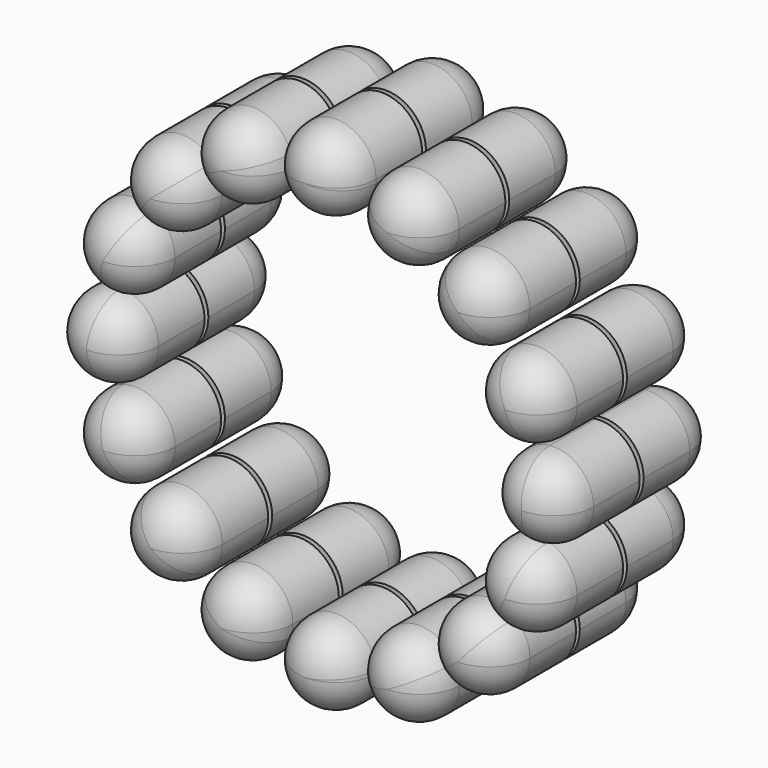
from build123d import *

# Parameters (mm, degrees)
F1_START      = 0.12
F1_DEPTH      = 4.88
F4_START      = -0.12
F4_DEPTH      = 4.88
F5_R          = 2
F5_2_R        = 2
F5_3_R        = 2
F5_4_R        = 2
F5_5_R        = 2
F5_6_R        = 2
F5_7_R        = 2
F5_8_R        = 2
F5_9_R        = 2
F5_10_R       = 2
F5_11_R       = 2
F5_12_R       = 2
F5_13_R       = 2
F5_14_R       = 2
F5_15_R       = 2
F5_16_R       = 2
F5_17_R       = 2
F5_18_R       = 2
F5_19_R       = 2
F5_20_R       = 2
F5_21_R       = 2
F5_22_R       = 2
F5_23_R       = 2
F5_24_R       = 2
F5_25_R       = 2
F5_26_R       = 2
F5_27_R       = 2
F5_28_R       = 2
F5_29_R       = 2
F5_30_R       = 2
F5_31_R       = 2
F5_32_R       = 2
F6_DEPTH      = 0.4
F6_DEPTH_BACK = 0.4


# Not quite as in the source:
# - the program builds the solid bodies; features that only make, move or delete a surface that nothing else refers to are left out


with BuildPart() as f1:
    # F0 (on Front) → F1 (new body)
    with BuildSketch(Plane.XZ.offset(F1_START)):
        with BuildLine():
            ThreePointArc((-1.9915265076, 10.691091954), (0, 8.875), (1.9915265076, 10.691091954))
            ThreePointArc((1.9915265076, 10.691091954), (1.8433395216, 10.717636139), (1.6947992849, 10.7421264368))
            ThreePointArc((1.6947992849, 10.7421264368), (0, 9.175), (-1.6947992849, 10.7421264368))
            ThreePointArc((-1.6947992849, 10.7421264368), (-1.8433395216, 10.717636139), (-1.9915265076, 10.691091954))
        make_face()
        with BuildLine():
            ThreePointArc((1.6947992849, 10.7421264368), (1.8433395216, 10.717636139), (1.9915265076, 10.691091954))
            ThreePointArc((1.9915265076, 10.691091954), (1.9978805038, 10.7829484255), (2, 10.875))
            ThreePointArc((2, 10.875), (-0.0920515745, 12.8728805038), (-1.9915265076, 10.691091954))
            ThreePointArc((-1.9915265076, 10.691091954), (-1.8433395216, 10.717636139), (-1.6947992849, 10.7421264368))
            ThreePointArc((-1.6947992849, 10.7421264368), (-0.0664876516, 12.5736993237), (1.7, 10.875))
            ThreePointArc((1.7, 10.875), (1.6986993237, 10.8085123484), (1.6947992849, 10.7421264368))
        make_face()
        with BuildLine():
            ThreePointArc((-1.6947992849, 10.7421264368), (0, 10.875), (1.6947992849, 10.7421264368))
            ThreePointArc((1.6947992849, 10.7421264368), (1.6986993237, 10.8085123484), (1.7, 10.875))
            ThreePointArc((1.7, 10.875), (-0.0664876516, 12.5736993237), (-1.6947992849, 10.7421264368))
        make_face()
        with BuildLine():
            ThreePointArc((-1.6947992849, 10.7421264368), (0, 9.175), (1.6947992849, 10.7421264368))
            ThreePointArc((1.6947992849, 10.7421264368), (0, 10.875), (-1.6947992849, 10.7421264368))
        make_face()
    extrude(amount=F1_DEPTH)

    # F5#3
    f5_3_edges = [f1.edges().sort_by_distance(p)[0] for p in [
        (-1.991527, -5, 11.058908),
    ]]
    fillet(f5_3_edges, radius=F5_3_R)


with BuildPart() as f1b:
    # F0 (on Front) → F1, piece 2 (new body)
    with BuildSketch(Plane.XZ.offset(F1_START)):
        with BuildLine():
            ThreePointArc((2.2513731858, 10.6394052361), (3.3963154622, 8.199430851), (5.9312343436, 9.1151568369))
            ThreePointArc((5.9312343436, 9.1151568369), (5.80448544, 9.1963891706), (5.6766241868, 9.2758591431))
            ThreePointArc((5.6766241868, 9.2758591431), (3.5111204919, 8.4765947108), (2.5450434447, 10.5730023581))
            ThreePointArc((2.5450434447, 10.5730023581), (2.3984381291, 10.6072201609), (2.2513731858, 10.6394052361))
        make_face()
        with BuildLine():
            ThreePointArc((5.6766241868, 9.2758591431), (5.80448544, 9.1963891706), (5.9312343436, 9.1151568369))
            ThreePointArc((5.9312343436, 9.1151568369), (6.1032157458, 9.5671399359), (6.161682327, 10.0471899161))
            ThreePointArc((6.161682327, 10.0471899161), (4.4611666485, 12.0246400775), (2.2513731858, 10.6394052361))
            ThreePointArc((2.2513731858, 10.6394052361), (2.3984381291, 10.6072201609), (2.5450434447, 10.5730023581))
            ThreePointArc((2.5450434447, 10.5730023581), (4.4278720151, 11.7262203059), (5.861682327, 10.0471899161))
            ThreePointArc((5.861682327, 10.0471899161), (5.8147705221, 9.650580008), (5.6766241868, 9.2758591431))
        make_face()
        with BuildLine():
            ThreePointArc((2.5450434447, 10.5730023581), (4.161682327, 10.0471899161), (5.6766241868, 9.2758591431))
            ThreePointArc((5.6766241868, 9.2758591431), (5.8147705221, 9.650580008), (5.861682327, 10.0471899161))
            ThreePointArc((5.861682327, 10.0471899161), (4.4278720151, 11.7262203059), (2.5450434447, 10.5730023581))
        make_face()
        with BuildLine():
            ThreePointArc((2.5450434447, 10.5730023581), (3.5111204919, 8.4765947108), (5.6766241868, 9.2758591431))
            ThreePointArc((5.6766241868, 9.2758591431), (4.161682327, 10.0471899161), (2.5450434447, 10.5730023581))
        make_face()
    extrude(amount=F1_DEPTH)

    # F5#4
    f5_4_edges = [f1b.edges().sort_by_distance(p)[0] for p in [
        (2.39213, -5, 10.979223),
    ]]
    fillet(f5_4_edges, radius=F5_4_R)


with BuildPart() as f1c:
    # F0 (on Front) → F1, piece 3 (new body)
    with BuildSketch(Plane.XZ.offset(F1_START)):
        with BuildLine():
            ThreePointArc((6.1515217205, 8.9679655174), (6.275572683, 6.275572683), (8.9679655174, 6.1515217205))
            ThreePointArc((8.9679655174, 6.1515217205), (8.8819510679, 6.2750753164), (8.7942345149, 6.3974263807))
            ThreePointArc((8.7942345149, 6.3974263807), (6.4877047174, 6.4877047174), (6.3974263807, 8.7942345149))
            ThreePointArc((6.3974263807, 8.7942345149), (6.2750753164, 8.8819510679), (6.1515217205, 8.9679655174))
        make_face()
        with BuildLine():
            ThreePointArc((8.7942345149, 6.3974263807), (8.8819510679, 6.2750753164), (8.9679655174, 6.1515217205))
            ThreePointArc((8.9679655174, 6.1515217205), (9.5003605388, 6.8401859112), (9.6897862454, 7.6897862454))
            ThreePointArc((9.6897862454, 7.6897862454), (8.3692974485, 9.5708137638), (6.1515217205, 8.9679655174))
            ThreePointArc((6.1515217205, 8.9679655174), (6.2750753164, 8.8819510679), (6.3974263807, 8.7942345149))
            ThreePointArc((6.3974263807, 8.7942345149), (8.2784237527, 9.2846235051), (9.3897862454, 7.6897862454))
            ThreePointArc((9.3897862454, 7.6897862454), (9.2337360597, 6.9782955772), (8.7942345149, 6.3974263807))
        make_face()
        with BuildLine():
            ThreePointArc((6.3974263807, 8.7942345149), (7.6897862454, 7.6897862454), (8.7942345149, 6.3974263807))
            ThreePointArc((8.7942345149, 6.3974263807), (9.2337360597, 6.9782955772), (9.3897862454, 7.6897862454))
            ThreePointArc((9.3897862454, 7.6897862454), (8.2784237527, 9.2846235051), (6.3974263807, 8.7942345149))
        make_face()
        with BuildLine():
            ThreePointArc((6.3974263807, 8.7942345149), (6.4877047174, 6.4877047174), (8.7942345149, 6.3974263807))
            ThreePointArc((8.7942345149, 6.3974263807), (7.6897862454, 7.6897862454), (6.3974263807, 8.7942345149))
        make_face()
    extrude(amount=F1_DEPTH)

    # F5#5
    f5_5_edges = [f1c.edges().sort_by_distance(p)[0] for p in [
        (6.411607, -5, 9.228051),
    ]]
    fillet(f5_5_edges, radius=F5_5_R)


with BuildPart() as f1d:
    # F0 (on Front) → F1, piece 4 (new body)
    with BuildSketch(Plane.XZ.offset(F1_START)):
        with BuildLine():
            ThreePointArc((9.1151568369, 5.9312343436), (8.199430851, 3.3963154622), (10.6394052361, 2.2513731858))
            ThreePointArc((10.6394052361, 2.2513731858), (10.6072201609, 2.3984381291), (10.5730023581, 2.5450434447))
            ThreePointArc((10.5730023581, 2.5450434447), (8.4765947108, 3.5111204919), (9.2758591431, 5.6766241868))
            ThreePointArc((9.2758591431, 5.6766241868), (9.1963891706, 5.80448544), (9.1151568369, 5.9312343436))
        make_face()
        with BuildLine():
            ThreePointArc((10.5730023581, 2.5450434447), (10.6072201609, 2.3984381291), (10.6394052361, 2.2513731858))
            ThreePointArc((10.6394052361, 2.2513731858), (11.6572257293, 2.975181303), (12.0471899161, 4.161682327))
            ThreePointArc((12.0471899161, 4.161682327), (11.0806147662, 5.8740003696), (9.1151568369, 5.9312343436))
            ThreePointArc((9.1151568369, 5.9312343436), (9.1963891706, 5.80448544), (9.2758591431, 5.6766241868))
            ThreePointArc((9.2758591431, 5.6766241868), (10.9356542333, 5.6110377551), (11.7471899161, 4.161682327))
            ThreePointArc((11.7471899161, 4.161682327), (11.422668224, 3.162653086), (10.5730023581, 2.5450434447))
        make_face()
        with BuildLine():
            ThreePointArc((9.2758591431, 5.6766241868), (10.0471899161, 4.161682327), (10.5730023581, 2.5450434447))
            ThreePointArc((10.5730023581, 2.5450434447), (11.422668224, 3.162653086), (11.7471899161, 4.161682327))
            ThreePointArc((11.7471899161, 4.161682327), (10.9356542333, 5.6110377551), (9.2758591431, 5.6766241868))
        make_face()
        with BuildLine():
            ThreePointArc((9.2758591431, 5.6766241868), (8.4765947108, 3.5111204919), (10.5730023581, 2.5450434447))
            ThreePointArc((10.5730023581, 2.5450434447), (10.0471899161, 4.161682327), (9.2758591431, 5.6766241868))
        make_face()
    extrude(amount=F1_DEPTH)

    # F5#6
    f5_6_edges = [f1d.edges().sort_by_distance(p)[0] for p in [
        (9.454975, -5, 6.071991),
    ]]
    fillet(f5_6_edges, radius=F5_6_R)


with BuildPart() as f1e:
    # F0 (on Front) → F1, piece 5 (new body)
    with BuildSketch(Plane.XZ.offset(F1_START)):
        with BuildLine():
            ThreePointArc((10.7421264368, -1.6947992849), (9.175, 0), (10.7421264368, 1.6947992849))
            ThreePointArc((10.7421264368, 1.6947992849), (10.717636139, 1.8433395216), (10.691091954, 1.9915265076))
            ThreePointArc((10.691091954, 1.9915265076), (8.875, 0), (10.691091954, -1.9915265076))
            ThreePointArc((10.691091954, -1.9915265076), (10.717636139, -1.8433395216), (10.7421264368, -1.6947992849))
        make_face()
        with BuildLine():
            ThreePointArc((10.691091954, 1.9915265076), (10.717636139, 1.8433395216), (10.7421264368, 1.6947992849))
            ThreePointArc((10.7421264368, 1.6947992849), (12.0291479417, 1.2481756802), (12.575, 0))
            ThreePointArc((12.575, 0), (12.0291479417, -1.2481756802), (10.7421264368, -1.6947992849))
            ThreePointArc((10.7421264368, -1.6947992849), (10.717636139, -1.8433395216), (10.691091954, -1.9915265076))
            ThreePointArc((10.691091954, -1.9915265076), (12.2226245597, -1.4778051448), (12.875, 0))
            ThreePointArc((12.875, 0), (12.2226245597, 1.4778051448), (10.691091954, 1.9915265076))
        make_face()
        with BuildLine():
            ThreePointArc((10.7421264368, 1.6947992849), (10.8417307198, 0.85), (10.875, 0))
            ThreePointArc((10.875, 0), (10.8417307198, -0.85), (10.7421264368, -1.6947992849))
            ThreePointArc((10.7421264368, -1.6947992849), (12.0291479417, -1.2481756802), (12.575, 0))
            ThreePointArc((12.575, 0), (12.0291479417, 1.2481756802), (10.7421264368, 1.6947992849))
        make_face()
        with BuildLine():
            ThreePointArc((10.7421264368, -1.6947992849), (10.8417307198, -0.85), (10.875, 0))
            ThreePointArc((10.875, 0), (10.8417307198, 0.85), (10.7421264368, 1.6947992849))
            ThreePointArc((10.7421264368, 1.6947992849), (9.175, 0), (10.7421264368, -1.6947992849))
        make_face()
    extrude(amount=F1_DEPTH)

    # F5#7
    f5_7_edges = [f1e.edges().sort_by_distance(p)[0] for p in [
        (11.058908, -5, 1.991527),
    ]]
    fillet(f5_7_edges, radius=F5_7_R)


with BuildPart() as f1f:
    # F0 (on Front) → F1, piece 6 (new body)
    with BuildSketch(Plane.XZ.offset(F1_START)):
        with BuildLine():
            ThreePointArc((10.5730023581, -2.5450434447), (10.6072201609, -2.3984381291), (10.6394052361, -2.2513731858))
            ThreePointArc((10.6394052361, -2.2513731858), (8.199430851, -3.3963154622), (9.1151568369, -5.9312343436))
            ThreePointArc((9.1151568369, -5.9312343436), (9.1963891706, -5.80448544), (9.2758591431, -5.6766241868))
            ThreePointArc((9.2758591431, -5.6766241868), (8.4765947108, -3.5111204919), (10.5730023581, -2.5450434447))
        make_face()
        with BuildLine():
            ThreePointArc((12.0471899161, -4.161682327), (11.6572257293, -2.975181303), (10.6394052361, -2.2513731858))
            ThreePointArc((10.6394052361, -2.2513731858), (10.6072201609, -2.3984381291), (10.5730023581, -2.5450434447))
            ThreePointArc((10.5730023581, -2.5450434447), (11.422668224, -3.162653086), (11.7471899161, -4.161682327))
            ThreePointArc((11.7471899161, -4.161682327), (10.9356542333, -5.6110377551), (9.2758591431, -5.6766241868))
            ThreePointArc((9.2758591431, -5.6766241868), (9.1963891706, -5.80448544), (9.1151568369, -5.9312343436))
            ThreePointArc((9.1151568369, -5.9312343436), (11.0806147662, -5.8740003696), (12.0471899161, -4.161682327))
        make_face()
        with BuildLine():
            ThreePointArc((11.7471899161, -4.161682327), (11.422668224, -3.162653086), (10.5730023581, -2.5450434447))
            ThreePointArc((10.5730023581, -2.5450434447), (10.0471899161, -4.161682327), (9.2758591431, -5.6766241868))
            ThreePointArc((9.2758591431, -5.6766241868), (10.9356542333, -5.6110377551), (11.7471899161, -4.161682327))
        make_face()
        with BuildLine():
            ThreePointArc((9.2758591431, -5.6766241868), (10.0471899161, -4.161682327), (10.5730023581, -2.5450434447))
            ThreePointArc((10.5730023581, -2.5450434447), (8.4765947108, -3.5111204919), (9.2758591431, -5.6766241868))
        make_face()
    extrude(amount=F1_DEPTH)

    # F5#8
    f5_8_edges = [f1f.edges().sort_by_distance(p)[0] for p in [
        (10.979223, -5, -2.39213),
    ]]
    fillet(f5_8_edges, radius=F5_8_R)


with BuildPart() as f1g:
    # F0 (on Front) → F1, piece 7 (new body)
    with BuildSketch(Plane.XZ.offset(F1_START)):
        with BuildLine():
            ThreePointArc((8.7942345149, -6.3974263807), (8.8819510679, -6.2750753164), (8.9679655174, -6.1515217205))
            ThreePointArc((8.9679655174, -6.1515217205), (6.275572683, -6.275572683), (6.1515217205, -8.9679655174))
            ThreePointArc((6.1515217205, -8.9679655174), (6.2750753164, -8.8819510679), (6.3974263807, -8.7942345149))
            ThreePointArc((6.3974263807, -8.7942345149), (6.4877047174, -6.4877047174), (8.7942345149, -6.3974263807))
        make_face()
        with BuildLine():
            ThreePointArc((9.6897862454, -7.6897862454), (9.5003605388, -6.8401859112), (8.9679655174, -6.1515217205))
            ThreePointArc((8.9679655174, -6.1515217205), (8.8819510679, -6.2750753164), (8.7942345149, -6.3974263807))
            ThreePointArc((8.7942345149, -6.3974263807), (9.2337360597, -6.9782955772), (9.3897862454, -7.6897862454))
            ThreePointArc((9.3897862454, -7.6897862454), (8.2784237527, -9.2846235051), (6.3974263807, -8.7942345149))
            ThreePointArc((6.3974263807, -8.7942345149), (6.2750753164, -8.8819510679), (6.1515217205, -8.9679655174))
            ThreePointArc((6.1515217205, -8.9679655174), (8.3692974485, -9.5708137638), (9.6897862454, -7.6897862454))
        make_face()
        with BuildLine():
            ThreePointArc((9.3897862454, -7.6897862454), (9.2337360597, -6.9782955772), (8.7942345149, -6.3974263807))
            ThreePointArc((8.7942345149, -6.3974263807), (7.6897862454, -7.6897862454), (6.3974263807, -8.7942345149))
            ThreePointArc((6.3974263807, -8.7942345149), (8.2784237527, -9.2846235051), (9.3897862454, -7.6897862454))
        make_face()
        with BuildLine():
            ThreePointArc((6.3974263807, -8.7942345149), (7.6897862454, -7.6897862454), (8.7942345149, -6.3974263807))
            ThreePointArc((8.7942345149, -6.3974263807), (6.4877047174, -6.4877047174), (6.3974263807, -8.7942345149))
        make_face()
    extrude(amount=F1_DEPTH)

    # F5#9
    f5_9_edges = [f1g.edges().sort_by_distance(p)[0] for p in [
        (9.228051, -5, -6.411607),
    ]]
    fillet(f5_9_edges, radius=F5_9_R)


with BuildPart() as f1h:
    # F0 (on Front) → F1, piece 8 (new body)
    with BuildSketch(Plane.XZ.offset(F1_START)):
        with BuildLine():
            ThreePointArc((5.6766241868, -9.2758591431), (5.80448544, -9.1963891706), (5.9312343436, -9.1151568369))
            ThreePointArc((5.9312343436, -9.1151568369), (3.3963154622, -8.199430851), (2.2513731858, -10.6394052361))
            ThreePointArc((2.2513731858, -10.6394052361), (2.3984381291, -10.6072201609), (2.5450434447, -10.5730023581))
            ThreePointArc((2.5450434447, -10.5730023581), (3.5111204919, -8.4765947108), (5.6766241868, -9.2758591431))
        make_face()
        with BuildLine():
            ThreePointArc((6.161682327, -10.0471899161), (6.1032157458, -9.5671399359), (5.9312343436, -9.1151568369))
            ThreePointArc((5.9312343436, -9.1151568369), (5.80448544, -9.1963891706), (5.6766241868, -9.2758591431))
            ThreePointArc((5.6766241868, -9.2758591431), (5.8147705221, -9.650580008), (5.861682327, -10.0471899161))
            ThreePointArc((5.861682327, -10.0471899161), (4.4278720151, -11.7262203059), (2.5450434447, -10.5730023581))
            ThreePointArc((2.5450434447, -10.5730023581), (2.3984381291, -10.6072201609), (2.2513731858, -10.6394052361))
            ThreePointArc((2.2513731858, -10.6394052361), (4.4611666485, -12.0246400775), (6.161682327, -10.0471899161))
        make_face()
        with BuildLine():
            ThreePointArc((5.861682327, -10.0471899161), (5.8147705221, -9.650580008), (5.6766241868, -9.2758591431))
            ThreePointArc((5.6766241868, -9.2758591431), (4.161682327, -10.0471899161), (2.5450434447, -10.5730023581))
            ThreePointArc((2.5450434447, -10.5730023581), (4.4278720151, -11.7262203059), (5.861682327, -10.0471899161))
        make_face()
        with BuildLine():
            ThreePointArc((2.5450434447, -10.5730023581), (4.161682327, -10.0471899161), (5.6766241868, -9.2758591431))
            ThreePointArc((5.6766241868, -9.2758591431), (3.5111204919, -8.4765947108), (2.5450434447, -10.5730023581))
        make_face()
    extrude(amount=F1_DEPTH)

    # F5#10
    f5_10_edges = [f1h.edges().sort_by_distance(p)[0] for p in [
        (6.071991, -5, -9.454975),
    ]]
    fillet(f5_10_edges, radius=F5_10_R)


with BuildPart() as f1i:
    # F0 (on Front) → F1, piece 9 (new body)
    with BuildSketch(Plane.XZ.offset(F1_START)):
        with BuildLine():
            ThreePointArc((1.6947992849, -10.7421264368), (1.8433395216, -10.717636139), (1.9915265076, -10.691091954))
            ThreePointArc((1.9915265076, -10.691091954), (0, -8.875), (-1.9915265076, -10.691091954))
            ThreePointArc((-1.9915265076, -10.691091954), (-1.8433395216, -10.717636139), (-1.6947992849, -10.7421264368))
            ThreePointArc((-1.6947992849, -10.7421264368), (0, -9.175), (1.6947992849, -10.7421264368))
        make_face()
        with BuildLine():
            ThreePointArc((2, -10.875), (1.9978805038, -10.7829484255), (1.9915265076, -10.691091954))
            ThreePointArc((1.9915265076, -10.691091954), (1.8433395216, -10.717636139), (1.6947992849, -10.7421264368))
            ThreePointArc((1.6947992849, -10.7421264368), (1.6986993237, -10.8085123484), (1.7, -10.875))
            ThreePointArc((1.7, -10.875), (-0.0664876516, -12.5736993237), (-1.6947992849, -10.7421264368))
            ThreePointArc((-1.6947992849, -10.7421264368), (-1.8433395216, -10.717636139), (-1.9915265076, -10.691091954))
            ThreePointArc((-1.9915265076, -10.691091954), (-0.0920515745, -12.8728805038), (2, -10.875))
        make_face()
        with BuildLine():
            ThreePointArc((1.7, -10.875), (1.6986993237, -10.8085123484), (1.6947992849, -10.7421264368))
            ThreePointArc((1.6947992849, -10.7421264368), (0, -10.875), (-1.6947992849, -10.7421264368))
            ThreePointArc((-1.6947992849, -10.7421264368), (-0.0664876516, -12.5736993237), (1.7, -10.875))
        make_face()
        with BuildLine():
            ThreePointArc((-1.6947992849, -10.7421264368), (0, -10.875), (1.6947992849, -10.7421264368))
            ThreePointArc((1.6947992849, -10.7421264368), (0, -9.175), (-1.6947992849, -10.7421264368))
        make_face()
    extrude(amount=F1_DEPTH)

    # F5#11
    f5_11_edges = [f1i.edges().sort_by_distance(p)[0] for p in [
        (1.991527, -5, -11.058908),
    ]]
    fillet(f5_11_edges, radius=F5_11_R)


with BuildPart() as f1j:
    # F0 (on Front) → F1, piece 10 (new body)
    with BuildSketch(Plane.XZ.offset(F1_START)):
        with BuildLine():
            ThreePointArc((-5.9312343436, -9.1151568369), (-4.9270491917, -11.8949489811), (-2.2513731858, -10.6394052361))
            ThreePointArc((-2.2513731858, -10.6394052361), (-2.3984381291, -10.6072201609), (-2.5450434447, -10.5730023581))
            ThreePointArc((-2.5450434447, -10.5730023581), (-4.812244162, -11.6177851213), (-5.6766241868, -9.2758591431))
            ThreePointArc((-5.6766241868, -9.2758591431), (-5.80448544, -9.1963891706), (-5.9312343436, -9.1151568369))
        make_face()
        with BuildLine():
            ThreePointArc((-2.5450434447, -10.5730023581), (-2.3984381291, -10.6072201609), (-2.2513731858, -10.6394052361))
            ThreePointArc((-2.2513731858, -10.6394052361), (-2.1842321655, -10.3466742376), (-2.161682327, -10.0471899161))
            ThreePointArc((-2.161682327, -10.0471899161), (-3.6816323468, -8.1056564972), (-5.9312343436, -9.1151568369))
            ThreePointArc((-5.9312343436, -9.1151568369), (-5.80448544, -9.1963891706), (-5.6766241868, -9.2758591431))
            ThreePointArc((-5.6766241868, -9.2758591431), (-3.7650724189, -8.3941017209), (-2.461682327, -10.0471899161))
            ThreePointArc((-2.461682327, -10.0471899161), (-2.4826519371, -10.3133796041), (-2.5450434447, -10.5730023581))
        make_face()
        with BuildLine():
            ThreePointArc((-5.6766241868, -9.2758591431), (-4.812244162, -11.6177851213), (-2.5450434447, -10.5730023581))
            ThreePointArc((-2.5450434447, -10.5730023581), (-4.161682327, -10.0471899161), (-5.6766241868, -9.2758591431))
        make_face()
        with BuildLine():
            ThreePointArc((-5.6766241868, -9.2758591431), (-4.161682327, -10.0471899161), (-2.5450434447, -10.5730023581))
            ThreePointArc((-2.5450434447, -10.5730023581), (-2.4826519371, -10.3133796041), (-2.461682327, -10.0471899161))
            ThreePointArc((-2.461682327, -10.0471899161), (-3.7650724189, -8.3941017209), (-5.6766241868, -9.2758591431))
        make_face()
    extrude(amount=F1_DEPTH)

    # F5#12
    f5_12_edges = [f1j.edges().sort_by_distance(p)[0] for p in [
        (-6.071991, -5, -9.454975),
    ]]
    fillet(f5_12_edges, radius=F5_12_R)


with BuildPart() as f1k:
    # F0 (on Front) → F1, piece 11 (new body)
    with BuildSketch(Plane.XZ.offset(F1_START)):
        with BuildLine():
            ThreePointArc((-8.9679655174, -6.1515217205), (-9.1039998078, -9.1039998078), (-6.1515217205, -8.9679655174))
            ThreePointArc((-6.1515217205, -8.9679655174), (-6.2750753164, -8.8819510679), (-6.3974263807, -8.7942345149))
            ThreePointArc((-6.3974263807, -8.7942345149), (-8.8918677734, -8.8918677734), (-8.7942345149, -6.3974263807))
            ThreePointArc((-8.7942345149, -6.3974263807), (-8.8819510679, -6.2750753164), (-8.9679655174, -6.1515217205))
        make_face()
        with BuildLine():
            ThreePointArc((-6.3974263807, -8.7942345149), (-6.2750753164, -8.8819510679), (-6.1515217205, -8.9679655174))
            ThreePointArc((-6.1515217205, -8.9679655174), (-5.808758727, -8.3692974485), (-5.6897862454, -7.6897862454))
            ThreePointArc((-5.6897862454, -7.6897862454), (-6.8401859112, -5.879211952), (-8.9679655174, -6.1515217205))
            ThreePointArc((-8.9679655174, -6.1515217205), (-8.8819510679, -6.2750753164), (-8.7942345149, -6.3974263807))
            ThreePointArc((-8.7942345149, -6.3974263807), (-6.9782955772, -6.1458364311), (-5.9897862454, -7.6897862454))
            ThreePointArc((-5.9897862454, -7.6897862454), (-6.0949489857, -8.2784237527), (-6.3974263807, -8.7942345149))
        make_face()
        with BuildLine():
            ThreePointArc((-8.7942345149, -6.3974263807), (-8.8918677734, -8.8918677734), (-6.3974263807, -8.7942345149))
            ThreePointArc((-6.3974263807, -8.7942345149), (-7.6897862454, -7.6897862454), (-8.7942345149, -6.3974263807))
        make_face()
        with BuildLine():
            ThreePointArc((-8.7942345149, -6.3974263807), (-7.6897862454, -7.6897862454), (-6.3974263807, -8.7942345149))
            ThreePointArc((-6.3974263807, -8.7942345149), (-6.0949489857, -8.2784237527), (-5.9897862454, -7.6897862454))
            ThreePointArc((-5.9897862454, -7.6897862454), (-6.9782955772, -6.1458364311), (-8.7942345149, -6.3974263807))
        make_face()
    extrude(amount=F1_DEPTH)

    # F5#13
    f5_13_edges = [f1k.edges().sort_by_distance(p)[0] for p in [
        (-9.228051, -5, -6.411607),
    ]]
    fillet(f5_13_edges, radius=F5_13_R)


with BuildPart() as f1l:
    # F0 (on Front) → F1, piece 12 (new body)
    with BuildSketch(Plane.XZ.offset(F1_START)):
        with BuildLine():
            ThreePointArc((-10.6394052361, -2.2513731858), (-11.8949489811, -4.9270491917), (-9.1151568369, -5.9312343436))
            ThreePointArc((-9.1151568369, -5.9312343436), (-9.1963891706, -5.80448544), (-9.2758591431, -5.6766241868))
            ThreePointArc((-9.2758591431, -5.6766241868), (-11.6177851213, -4.812244162), (-10.5730023581, -2.5450434447))
            ThreePointArc((-10.5730023581, -2.5450434447), (-10.6072201609, -2.3984381291), (-10.6394052361, -2.2513731858))
        make_face()
        with BuildLine():
            ThreePointArc((-9.2758591431, -5.6766241868), (-9.1963891706, -5.80448544), (-9.1151568369, -5.9312343436))
            ThreePointArc((-9.1151568369, -5.9312343436), (-8.3348718734, -5.1951071771), (-8.0471899161, -4.161682327))
            ThreePointArc((-8.0471899161, -4.161682327), (-8.8606888921, -2.5516465137), (-10.6394052361, -2.2513731858))
            ThreePointArc((-10.6394052361, -2.2513731858), (-10.6072201609, -2.3984381291), (-10.5730023581, -2.5450434447))
            ThreePointArc((-10.5730023581, -2.5450434447), (-9.0481606751, -2.786204019), (-8.3471899161, -4.161682327))
            ThreePointArc((-8.3471899161, -4.161682327), (-8.5978344879, -5.0501466442), (-9.2758591431, -5.6766241868))
        make_face()
        with BuildLine():
            ThreePointArc((-10.5730023581, -2.5450434447), (-11.6177851213, -4.812244162), (-9.2758591431, -5.6766241868))
            ThreePointArc((-9.2758591431, -5.6766241868), (-10.0471899161, -4.161682327), (-10.5730023581, -2.5450434447))
        make_face()
        with BuildLine():
            ThreePointArc((-10.5730023581, -2.5450434447), (-10.0471899161, -4.161682327), (-9.2758591431, -5.6766241868))
            ThreePointArc((-9.2758591431, -5.6766241868), (-8.5978344879, -5.0501466442), (-8.3471899161, -4.161682327))
            ThreePointArc((-8.3471899161, -4.161682327), (-9.0481606751, -2.786204019), (-10.5730023581, -2.5450434447))
        make_face()
    extrude(amount=F1_DEPTH)

    # F5#14
    f5_14_edges = [f1l.edges().sort_by_distance(p)[0] for p in [
        (-10.979223, -5, -2.39213),
    ]]
    fillet(f5_14_edges, radius=F5_14_R)


with BuildPart() as f1m:
    # F0 (on Front) → F1, piece 13 (new body)
    with BuildSketch(Plane.XZ.offset(F1_START)):
        with BuildLine():
            ThreePointArc((-10.7421264368, 1.6947992849), (-10.717636139, 1.8433395216), (-10.691091954, 1.9915265076))
            ThreePointArc((-10.691091954, 1.9915265076), (-12.875, 0), (-10.691091954, -1.9915265076))
            ThreePointArc((-10.691091954, -1.9915265076), (-10.717636139, -1.8433395216), (-10.7421264368, -1.6947992849))
            ThreePointArc((-10.7421264368, -1.6947992849), (-12.575, 0), (-10.7421264368, 1.6947992849))
        make_face()
        with BuildLine():
            ThreePointArc((-8.875, 0), (-9.3971948552, 1.3476245597), (-10.691091954, 1.9915265076))
            ThreePointArc((-10.691091954, 1.9915265076), (-10.717636139, 1.8433395216), (-10.7421264368, 1.6947992849))
            ThreePointArc((-10.7421264368, 1.6947992849), (-9.6268243198, 1.1541479417), (-9.175, 0))
            ThreePointArc((-9.175, 0), (-9.6268243198, -1.1541479417), (-10.7421264368, -1.6947992849))
            ThreePointArc((-10.7421264368, -1.6947992849), (-10.717636139, -1.8433395216), (-10.691091954, -1.9915265076))
            ThreePointArc((-10.691091954, -1.9915265076), (-9.3971948552, -1.3476245597), (-8.875, 0))
        make_face()
        with BuildLine():
            ThreePointArc((-10.7421264368, -1.6947992849), (-10.875, 0), (-10.7421264368, 1.6947992849))
            ThreePointArc((-10.7421264368, 1.6947992849), (-12.575, 0), (-10.7421264368, -1.6947992849))
        make_face()
        with BuildLine():
            ThreePointArc((-9.175, 0), (-9.6268243198, 1.1541479417), (-10.7421264368, 1.6947992849))
            ThreePointArc((-10.7421264368, 1.6947992849), (-10.875, 0), (-10.7421264368, -1.6947992849))
            ThreePointArc((-10.7421264368, -1.6947992849), (-9.6268243198, -1.1541479417), (-9.175, 0))
        make_face()
    extrude(amount=F1_DEPTH)

    # F5#15
    f5_15_edges = [f1m.edges().sort_by_distance(p)[0] for p in [
        (-11.058908, -5, 1.991527),
    ]]
    fillet(f5_15_edges, radius=F5_15_R)


with BuildPart() as f1n:
    # F0 (on Front) → F1, piece 14 (new body)
    with BuildSketch(Plane.XZ.offset(F1_START)):
        with BuildLine():
            ThreePointArc((-9.2758591431, 5.6766241868), (-9.1963891706, 5.80448544), (-9.1151568369, 5.9312343436))
            ThreePointArc((-9.1151568369, 5.9312343436), (-11.8949489811, 4.9270491917), (-10.6394052361, 2.2513731858))
            ThreePointArc((-10.6394052361, 2.2513731858), (-10.6072201609, 2.3984381291), (-10.5730023581, 2.5450434447))
            ThreePointArc((-10.5730023581, 2.5450434447), (-11.6177851213, 4.812244162), (-9.2758591431, 5.6766241868))
        make_face()
        with BuildLine():
            ThreePointArc((-8.0471899161, 4.161682327), (-8.3348718734, 5.1951071771), (-9.1151568369, 5.9312343436))
            ThreePointArc((-9.1151568369, 5.9312343436), (-9.1963891706, 5.80448544), (-9.2758591431, 5.6766241868))
            ThreePointArc((-9.2758591431, 5.6766241868), (-8.5978344879, 5.0501466442), (-8.3471899161, 4.161682327))
            ThreePointArc((-8.3471899161, 4.161682327), (-9.0481606751, 2.786204019), (-10.5730023581, 2.5450434447))
            ThreePointArc((-10.5730023581, 2.5450434447), (-10.6072201609, 2.3984381291), (-10.6394052361, 2.2513731858))
            ThreePointArc((-10.6394052361, 2.2513731858), (-8.8606888921, 2.5516465137), (-8.0471899161, 4.161682327))
        make_face()
        with BuildLine():
            ThreePointArc((-10.5730023581, 2.5450434447), (-10.0471899161, 4.161682327), (-9.2758591431, 5.6766241868))
            ThreePointArc((-9.2758591431, 5.6766241868), (-11.6177851213, 4.812244162), (-10.5730023581, 2.5450434447))
        make_face()
        with BuildLine():
            ThreePointArc((-8.3471899161, 4.161682327), (-8.5978344879, 5.0501466442), (-9.2758591431, 5.6766241868))
            ThreePointArc((-9.2758591431, 5.6766241868), (-10.0471899161, 4.161682327), (-10.5730023581, 2.5450434447))
            ThreePointArc((-10.5730023581, 2.5450434447), (-9.0481606751, 2.786204019), (-8.3471899161, 4.161682327))
        make_face()
    extrude(amount=F1_DEPTH)

    # F5#16
    f5_16_edges = [f1n.edges().sort_by_distance(p)[0] for p in [
        (-9.454975, -5, 6.071991),
    ]]
    fillet(f5_16_edges, radius=F5_16_R)


with BuildPart() as f1o:
    # F0 (on Front) → F1, piece 15 (new body)
    with BuildSketch(Plane.XZ.offset(F1_START)):
        with BuildLine():
            ThreePointArc((-6.3974263807, 8.7942345149), (-6.2750753164, 8.8819510679), (-6.1515217205, 8.9679655174))
            ThreePointArc((-6.1515217205, 8.9679655174), (-9.1039998078, 9.1039998078), (-8.9679655174, 6.1515217205))
            ThreePointArc((-8.9679655174, 6.1515217205), (-8.8819510679, 6.2750753164), (-8.7942345149, 6.3974263807))
            ThreePointArc((-8.7942345149, 6.3974263807), (-8.8918677734, 8.8918677734), (-6.3974263807, 8.7942345149))
        make_face()
        with BuildLine():
            ThreePointArc((-5.6897862454, 7.6897862454), (-5.808758727, 8.3692974485), (-6.1515217205, 8.9679655174))
            ThreePointArc((-6.1515217205, 8.9679655174), (-6.2750753164, 8.8819510679), (-6.3974263807, 8.7942345149))
            ThreePointArc((-6.3974263807, 8.7942345149), (-6.0949489857, 8.2784237527), (-5.9897862454, 7.6897862454))
            ThreePointArc((-5.9897862454, 7.6897862454), (-6.9782955772, 6.1458364311), (-8.7942345149, 6.3974263807))
            ThreePointArc((-8.7942345149, 6.3974263807), (-8.8819510679, 6.2750753164), (-8.9679655174, 6.1515217205))
            ThreePointArc((-8.9679655174, 6.1515217205), (-6.8401859112, 5.879211952), (-5.6897862454, 7.6897862454))
        make_face()
        with BuildLine():
            ThreePointArc((-8.7942345149, 6.3974263807), (-7.6897862454, 7.6897862454), (-6.3974263807, 8.7942345149))
            ThreePointArc((-6.3974263807, 8.7942345149), (-8.8918677734, 8.8918677734), (-8.7942345149, 6.3974263807))
        make_face()
        with BuildLine():
            ThreePointArc((-5.9897862454, 7.6897862454), (-6.0949489857, 8.2784237527), (-6.3974263807, 8.7942345149))
            ThreePointArc((-6.3974263807, 8.7942345149), (-7.6897862454, 7.6897862454), (-8.7942345149, 6.3974263807))
            ThreePointArc((-8.7942345149, 6.3974263807), (-6.9782955772, 6.1458364311), (-5.9897862454, 7.6897862454))
        make_face()
    extrude(amount=F1_DEPTH)

    # F5
    f5_edges = [f1o.edges().sort_by_distance(p)[0] for p in [
        (-6.411607, -5, 9.228051),
    ]]
    fillet(f5_edges, radius=F5_R)


with BuildPart() as f1p:
    # F0 (on Front) → F1, piece 16 (new body)
    with BuildSketch(Plane.XZ.offset(F1_START)):
        with BuildLine():
            ThreePointArc((-2.5450434447, 10.5730023581), (-2.3984381291, 10.6072201609), (-2.2513731858, 10.6394052361))
            ThreePointArc((-2.2513731858, 10.6394052361), (-4.9270491917, 11.8949489811), (-5.9312343436, 9.1151568369))
            ThreePointArc((-5.9312343436, 9.1151568369), (-5.80448544, 9.1963891706), (-5.6766241868, 9.2758591431))
            ThreePointArc((-5.6766241868, 9.2758591431), (-4.812244162, 11.6177851213), (-2.5450434447, 10.5730023581))
        make_face()
        with BuildLine():
            ThreePointArc((-2.161682327, 10.0471899161), (-2.1842321655, 10.3466742376), (-2.2513731858, 10.6394052361))
            ThreePointArc((-2.2513731858, 10.6394052361), (-2.3984381291, 10.6072201609), (-2.5450434447, 10.5730023581))
            ThreePointArc((-2.5450434447, 10.5730023581), (-2.4826519371, 10.3133796041), (-2.461682327, 10.0471899161))
            ThreePointArc((-2.461682327, 10.0471899161), (-3.7650724189, 8.3941017209), (-5.6766241868, 9.2758591431))
            ThreePointArc((-5.6766241868, 9.2758591431), (-5.80448544, 9.1963891706), (-5.9312343436, 9.1151568369))
            ThreePointArc((-5.9312343436, 9.1151568369), (-3.6816323468, 8.1056564972), (-2.161682327, 10.0471899161))
        make_face()
        with BuildLine():
            ThreePointArc((-5.6766241868, 9.2758591431), (-4.161682327, 10.0471899161), (-2.5450434447, 10.5730023581))
            ThreePointArc((-2.5450434447, 10.5730023581), (-4.812244162, 11.6177851213), (-5.6766241868, 9.2758591431))
        make_face()
        with BuildLine():
            ThreePointArc((-2.461682327, 10.0471899161), (-2.4826519371, 10.3133796041), (-2.5450434447, 10.5730023581))
            ThreePointArc((-2.5450434447, 10.5730023581), (-4.161682327, 10.0471899161), (-5.6766241868, 9.2758591431))
            ThreePointArc((-5.6766241868, 9.2758591431), (-3.7650724189, 8.3941017209), (-2.461682327, 10.0471899161))
        make_face()
    extrude(amount=F1_DEPTH)

    # F5#2
    f5_2_edges = [f1p.edges().sort_by_distance(p)[0] for p in [
        (-2.39213, -5, 10.979223),
    ]]
    fillet(f5_2_edges, radius=F5_2_R)


with BuildPart() as f4:
    # F0 (on Front) → F4 (new body)
    with BuildSketch(Plane.XZ.offset(F4_START)):
        with BuildLine():
            ThreePointArc((11.7471899161, -4.161682327), (11.422668224, -3.162653086), (10.5730023581, -2.5450434447))
            ThreePointArc((10.5730023581, -2.5450434447), (10.0471899161, -4.161682327), (9.2758591431, -5.6766241868))
            ThreePointArc((9.2758591431, -5.6766241868), (10.9356542333, -5.6110377551), (11.7471899161, -4.161682327))
        make_face()
        with BuildLine():
            ThreePointArc((12.0471899161, -4.161682327), (11.6572257293, -2.975181303), (10.6394052361, -2.2513731858))
            ThreePointArc((10.6394052361, -2.2513731858), (10.6072201609, -2.3984381291), (10.5730023581, -2.5450434447))
            ThreePointArc((10.5730023581, -2.5450434447), (11.422668224, -3.162653086), (11.7471899161, -4.161682327))
            ThreePointArc((11.7471899161, -4.161682327), (10.9356542333, -5.6110377551), (9.2758591431, -5.6766241868))
            ThreePointArc((9.2758591431, -5.6766241868), (9.1963891706, -5.80448544), (9.1151568369, -5.9312343436))
            ThreePointArc((9.1151568369, -5.9312343436), (11.0806147662, -5.8740003696), (12.0471899161, -4.161682327))
        make_face()
        with BuildLine():
            ThreePointArc((9.2758591431, -5.6766241868), (10.0471899161, -4.161682327), (10.5730023581, -2.5450434447))
            ThreePointArc((10.5730023581, -2.5450434447), (8.4765947108, -3.5111204919), (9.2758591431, -5.6766241868))
        make_face()
        with BuildLine():
            ThreePointArc((10.5730023581, -2.5450434447), (10.6072201609, -2.3984381291), (10.6394052361, -2.2513731858))
            ThreePointArc((10.6394052361, -2.2513731858), (8.199430851, -3.3963154622), (9.1151568369, -5.9312343436))
            ThreePointArc((9.1151568369, -5.9312343436), (9.1963891706, -5.80448544), (9.2758591431, -5.6766241868))
            ThreePointArc((9.2758591431, -5.6766241868), (8.4765947108, -3.5111204919), (10.5730023581, -2.5450434447))
        make_face()
    extrude(amount=-F4_DEPTH)

    # F5#29
    f5_29_edges = [f4.edges().sort_by_distance(p)[0] for p in [
        (9.454975, 5, -6.071991),
    ]]
    fillet(f5_29_edges, radius=F5_29_R)


with BuildPart() as f4b:
    # F0 (on Front) → F4, piece 2 (new body)
    with BuildSketch(Plane.XZ.offset(F4_START)):
        with BuildLine():
            ThreePointArc((8.7942345149, -6.3974263807), (8.8819510679, -6.2750753164), (8.9679655174, -6.1515217205))
            ThreePointArc((8.9679655174, -6.1515217205), (6.275572683, -6.275572683), (6.1515217205, -8.9679655174))
            ThreePointArc((6.1515217205, -8.9679655174), (6.2750753164, -8.8819510679), (6.3974263807, -8.7942345149))
            ThreePointArc((6.3974263807, -8.7942345149), (6.4877047174, -6.4877047174), (8.7942345149, -6.3974263807))
        make_face()
        with BuildLine():
            ThreePointArc((6.3974263807, -8.7942345149), (7.6897862454, -7.6897862454), (8.7942345149, -6.3974263807))
            ThreePointArc((8.7942345149, -6.3974263807), (6.4877047174, -6.4877047174), (6.3974263807, -8.7942345149))
        make_face()
        with BuildLine():
            ThreePointArc((9.3897862454, -7.6897862454), (9.2337360597, -6.9782955772), (8.7942345149, -6.3974263807))
            ThreePointArc((8.7942345149, -6.3974263807), (7.6897862454, -7.6897862454), (6.3974263807, -8.7942345149))
            ThreePointArc((6.3974263807, -8.7942345149), (8.2784237527, -9.2846235051), (9.3897862454, -7.6897862454))
        make_face()
        with BuildLine():
            ThreePointArc((9.6897862454, -7.6897862454), (9.5003605388, -6.8401859112), (8.9679655174, -6.1515217205))
            ThreePointArc((8.9679655174, -6.1515217205), (8.8819510679, -6.2750753164), (8.7942345149, -6.3974263807))
            ThreePointArc((8.7942345149, -6.3974263807), (9.2337360597, -6.9782955772), (9.3897862454, -7.6897862454))
            ThreePointArc((9.3897862454, -7.6897862454), (8.2784237527, -9.2846235051), (6.3974263807, -8.7942345149))
            ThreePointArc((6.3974263807, -8.7942345149), (6.2750753164, -8.8819510679), (6.1515217205, -8.9679655174))
            ThreePointArc((6.1515217205, -8.9679655174), (8.3692974485, -9.5708137638), (9.6897862454, -7.6897862454))
        make_face()
    extrude(amount=-F4_DEPTH)

    # F5#28
    f5_28_edges = [f4b.edges().sort_by_distance(p)[0] for p in [
        (9.228051, 5, -6.411607),
    ]]
    fillet(f5_28_edges, radius=F5_28_R)


with BuildPart() as f4c:
    # F0 (on Front) → F4, piece 3 (new body)
    with BuildSketch(Plane.XZ.offset(F4_START)):
        with BuildLine():
            ThreePointArc((6.161682327, -10.0471899161), (6.1032157458, -9.5671399359), (5.9312343436, -9.1151568369))
            ThreePointArc((5.9312343436, -9.1151568369), (5.80448544, -9.1963891706), (5.6766241868, -9.2758591431))
            ThreePointArc((5.6766241868, -9.2758591431), (5.8147705221, -9.650580008), (5.861682327, -10.0471899161))
            ThreePointArc((5.861682327, -10.0471899161), (4.4278720151, -11.7262203059), (2.5450434447, -10.5730023581))
            ThreePointArc((2.5450434447, -10.5730023581), (2.3984381291, -10.6072201609), (2.2513731858, -10.6394052361))
            ThreePointArc((2.2513731858, -10.6394052361), (4.4611666485, -12.0246400775), (6.161682327, -10.0471899161))
        make_face()
        with BuildLine():
            ThreePointArc((5.861682327, -10.0471899161), (5.8147705221, -9.650580008), (5.6766241868, -9.2758591431))
            ThreePointArc((5.6766241868, -9.2758591431), (4.161682327, -10.0471899161), (2.5450434447, -10.5730023581))
            ThreePointArc((2.5450434447, -10.5730023581), (4.4278720151, -11.7262203059), (5.861682327, -10.0471899161))
        make_face()
        with BuildLine():
            ThreePointArc((2.5450434447, -10.5730023581), (4.161682327, -10.0471899161), (5.6766241868, -9.2758591431))
            ThreePointArc((5.6766241868, -9.2758591431), (3.5111204919, -8.4765947108), (2.5450434447, -10.5730023581))
        make_face()
        with BuildLine():
            ThreePointArc((5.6766241868, -9.2758591431), (5.80448544, -9.1963891706), (5.9312343436, -9.1151568369))
            ThreePointArc((5.9312343436, -9.1151568369), (3.3963154622, -8.199430851), (2.2513731858, -10.6394052361))
            ThreePointArc((2.2513731858, -10.6394052361), (2.3984381291, -10.6072201609), (2.5450434447, -10.5730023581))
            ThreePointArc((2.5450434447, -10.5730023581), (3.5111204919, -8.4765947108), (5.6766241868, -9.2758591431))
        make_face()
    extrude(amount=-F4_DEPTH)

    # F5#27
    f5_27_edges = [f4c.edges().sort_by_distance(p)[0] for p in [
        (2.39213, 5, -10.979223),
    ]]
    fillet(f5_27_edges, radius=F5_27_R)


with BuildPart() as f4d:
    # F0 (on Front) → F4, piece 4 (new body)
    with BuildSketch(Plane.XZ.offset(F4_START)):
        with BuildLine():
            ThreePointArc((-1.6947992849, -10.7421264368), (0, -10.875), (1.6947992849, -10.7421264368))
            ThreePointArc((1.6947992849, -10.7421264368), (0, -9.175), (-1.6947992849, -10.7421264368))
        make_face()
        with BuildLine():
            ThreePointArc((1.7, -10.875), (1.6986993237, -10.8085123484), (1.6947992849, -10.7421264368))
            ThreePointArc((1.6947992849, -10.7421264368), (0, -10.875), (-1.6947992849, -10.7421264368))
            ThreePointArc((-1.6947992849, -10.7421264368), (-0.0664876516, -12.5736993237), (1.7, -10.875))
        make_face()
        with BuildLine():
            ThreePointArc((2, -10.875), (1.9978805038, -10.7829484255), (1.9915265076, -10.691091954))
            ThreePointArc((1.9915265076, -10.691091954), (1.8433395216, -10.717636139), (1.6947992849, -10.7421264368))
            ThreePointArc((1.6947992849, -10.7421264368), (1.6986993237, -10.8085123484), (1.7, -10.875))
            ThreePointArc((1.7, -10.875), (-0.0664876516, -12.5736993237), (-1.6947992849, -10.7421264368))
            ThreePointArc((-1.6947992849, -10.7421264368), (-1.8433395216, -10.717636139), (-1.9915265076, -10.691091954))
            ThreePointArc((-1.9915265076, -10.691091954), (-0.0920515745, -12.8728805038), (2, -10.875))
        make_face()
        with BuildLine():
            ThreePointArc((1.6947992849, -10.7421264368), (1.8433395216, -10.717636139), (1.9915265076, -10.691091954))
            ThreePointArc((1.9915265076, -10.691091954), (0, -8.875), (-1.9915265076, -10.691091954))
            ThreePointArc((-1.9915265076, -10.691091954), (-1.8433395216, -10.717636139), (-1.6947992849, -10.7421264368))
            ThreePointArc((-1.6947992849, -10.7421264368), (0, -9.175), (1.6947992849, -10.7421264368))
        make_face()
    extrude(amount=-F4_DEPTH)

    # F5#26
    f5_26_edges = [f4d.edges().sort_by_distance(p)[0] for p in [
        (-1.991527, 5, -11.058908),
    ]]
    fillet(f5_26_edges, radius=F5_26_R)


with BuildPart() as f4e:
    # F0 (on Front) → F4, piece 5 (new body)
    with BuildSketch(Plane.XZ.offset(F4_START)):
        with BuildLine():
            ThreePointArc((-2.5450434447, -10.5730023581), (-2.3984381291, -10.6072201609), (-2.2513731858, -10.6394052361))
            ThreePointArc((-2.2513731858, -10.6394052361), (-2.1842321655, -10.3466742376), (-2.161682327, -10.0471899161))
            ThreePointArc((-2.161682327, -10.0471899161), (-3.6816323468, -8.1056564972), (-5.9312343436, -9.1151568369))
            ThreePointArc((-5.9312343436, -9.1151568369), (-5.80448544, -9.1963891706), (-5.6766241868, -9.2758591431))
            ThreePointArc((-5.6766241868, -9.2758591431), (-3.7650724189, -8.3941017209), (-2.461682327, -10.0471899161))
            ThreePointArc((-2.461682327, -10.0471899161), (-2.4826519371, -10.3133796041), (-2.5450434447, -10.5730023581))
        make_face()
        with BuildLine():
            ThreePointArc((-5.6766241868, -9.2758591431), (-4.161682327, -10.0471899161), (-2.5450434447, -10.5730023581))
            ThreePointArc((-2.5450434447, -10.5730023581), (-2.4826519371, -10.3133796041), (-2.461682327, -10.0471899161))
            ThreePointArc((-2.461682327, -10.0471899161), (-3.7650724189, -8.3941017209), (-5.6766241868, -9.2758591431))
        make_face()
        with BuildLine():
            ThreePointArc((-5.6766241868, -9.2758591431), (-4.812244162, -11.6177851213), (-2.5450434447, -10.5730023581))
            ThreePointArc((-2.5450434447, -10.5730023581), (-4.161682327, -10.0471899161), (-5.6766241868, -9.2758591431))
        make_face()
        with BuildLine():
            ThreePointArc((-5.9312343436, -9.1151568369), (-4.9270491917, -11.8949489811), (-2.2513731858, -10.6394052361))
            ThreePointArc((-2.2513731858, -10.6394052361), (-2.3984381291, -10.6072201609), (-2.5450434447, -10.5730023581))
            ThreePointArc((-2.5450434447, -10.5730023581), (-4.812244162, -11.6177851213), (-5.6766241868, -9.2758591431))
            ThreePointArc((-5.6766241868, -9.2758591431), (-5.80448544, -9.1963891706), (-5.9312343436, -9.1151568369))
        make_face()
    extrude(amount=-F4_DEPTH)

    # F5#25
    f5_25_edges = [f4e.edges().sort_by_distance(p)[0] for p in [
        (-2.39213, 5, -10.979223),
    ]]
    fillet(f5_25_edges, radius=F5_25_R)


with BuildPart() as f4f:
    # F0 (on Front) → F4, piece 6 (new body)
    with BuildSketch(Plane.XZ.offset(F4_START)):
        with BuildLine():
            ThreePointArc((-8.9679655174, -6.1515217205), (-9.1039998078, -9.1039998078), (-6.1515217205, -8.9679655174))
            ThreePointArc((-6.1515217205, -8.9679655174), (-6.2750753164, -8.8819510679), (-6.3974263807, -8.7942345149))
            ThreePointArc((-6.3974263807, -8.7942345149), (-8.8918677734, -8.8918677734), (-8.7942345149, -6.3974263807))
            ThreePointArc((-8.7942345149, -6.3974263807), (-8.8819510679, -6.2750753164), (-8.9679655174, -6.1515217205))
        make_face()
        with BuildLine():
            ThreePointArc((-8.7942345149, -6.3974263807), (-8.8918677734, -8.8918677734), (-6.3974263807, -8.7942345149))
            ThreePointArc((-6.3974263807, -8.7942345149), (-7.6897862454, -7.6897862454), (-8.7942345149, -6.3974263807))
        make_face()
        with BuildLine():
            ThreePointArc((-8.7942345149, -6.3974263807), (-7.6897862454, -7.6897862454), (-6.3974263807, -8.7942345149))
            ThreePointArc((-6.3974263807, -8.7942345149), (-6.0949489857, -8.2784237527), (-5.9897862454, -7.6897862454))
            ThreePointArc((-5.9897862454, -7.6897862454), (-6.9782955772, -6.1458364311), (-8.7942345149, -6.3974263807))
        make_face()
        with BuildLine():
            ThreePointArc((-6.3974263807, -8.7942345149), (-6.2750753164, -8.8819510679), (-6.1515217205, -8.9679655174))
            ThreePointArc((-6.1515217205, -8.9679655174), (-5.808758727, -8.3692974485), (-5.6897862454, -7.6897862454))
            ThreePointArc((-5.6897862454, -7.6897862454), (-6.8401859112, -5.879211952), (-8.9679655174, -6.1515217205))
            ThreePointArc((-8.9679655174, -6.1515217205), (-8.8819510679, -6.2750753164), (-8.7942345149, -6.3974263807))
            ThreePointArc((-8.7942345149, -6.3974263807), (-6.9782955772, -6.1458364311), (-5.9897862454, -7.6897862454))
            ThreePointArc((-5.9897862454, -7.6897862454), (-6.0949489857, -8.2784237527), (-6.3974263807, -8.7942345149))
        make_face()
    extrude(amount=-F4_DEPTH)

    # F5#24
    f5_24_edges = [f4f.edges().sort_by_distance(p)[0] for p in [
        (-9.228051, 5, -6.411607),
    ]]
    fillet(f5_24_edges, radius=F5_24_R)


with BuildPart() as f4g:
    # F0 (on Front) → F4, piece 7 (new body)
    with BuildSketch(Plane.XZ.offset(F4_START)):
        with BuildLine():
            ThreePointArc((-10.5730023581, -2.5450434447), (-10.0471899161, -4.161682327), (-9.2758591431, -5.6766241868))
            ThreePointArc((-9.2758591431, -5.6766241868), (-8.5978344879, -5.0501466442), (-8.3471899161, -4.161682327))
            ThreePointArc((-8.3471899161, -4.161682327), (-9.0481606751, -2.786204019), (-10.5730023581, -2.5450434447))
        make_face()
        with BuildLine():
            ThreePointArc((-9.2758591431, -5.6766241868), (-9.1963891706, -5.80448544), (-9.1151568369, -5.9312343436))
            ThreePointArc((-9.1151568369, -5.9312343436), (-8.3348718734, -5.1951071771), (-8.0471899161, -4.161682327))
            ThreePointArc((-8.0471899161, -4.161682327), (-8.8606888921, -2.5516465137), (-10.6394052361, -2.2513731858))
            ThreePointArc((-10.6394052361, -2.2513731858), (-10.6072201609, -2.3984381291), (-10.5730023581, -2.5450434447))
            ThreePointArc((-10.5730023581, -2.5450434447), (-9.0481606751, -2.786204019), (-8.3471899161, -4.161682327))
            ThreePointArc((-8.3471899161, -4.161682327), (-8.5978344879, -5.0501466442), (-9.2758591431, -5.6766241868))
        make_face()
        with BuildLine():
            ThreePointArc((-10.5730023581, -2.5450434447), (-11.6177851213, -4.812244162), (-9.2758591431, -5.6766241868))
            ThreePointArc((-9.2758591431, -5.6766241868), (-10.0471899161, -4.161682327), (-10.5730023581, -2.5450434447))
        make_face()
        with BuildLine():
            ThreePointArc((-10.6394052361, -2.2513731858), (-11.8949489811, -4.9270491917), (-9.1151568369, -5.9312343436))
            ThreePointArc((-9.1151568369, -5.9312343436), (-9.1963891706, -5.80448544), (-9.2758591431, -5.6766241868))
            ThreePointArc((-9.2758591431, -5.6766241868), (-11.6177851213, -4.812244162), (-10.5730023581, -2.5450434447))
            ThreePointArc((-10.5730023581, -2.5450434447), (-10.6072201609, -2.3984381291), (-10.6394052361, -2.2513731858))
        make_face()
    extrude(amount=-F4_DEPTH)

    # F5#23
    f5_23_edges = [f4g.edges().sort_by_distance(p)[0] for p in [
        (-9.454975, 5, -6.071991),
    ]]
    fillet(f5_23_edges, radius=F5_23_R)


with BuildPart() as f4h:
    # F0 (on Front) → F4, piece 8 (new body)
    with BuildSketch(Plane.XZ.offset(F4_START)):
        with BuildLine():
            ThreePointArc((-10.7421264368, 1.6947992849), (-10.717636139, 1.8433395216), (-10.691091954, 1.9915265076))
            ThreePointArc((-10.691091954, 1.9915265076), (-12.875, 0), (-10.691091954, -1.9915265076))
            ThreePointArc((-10.691091954, -1.9915265076), (-10.717636139, -1.8433395216), (-10.7421264368, -1.6947992849))
            ThreePointArc((-10.7421264368, -1.6947992849), (-12.575, 0), (-10.7421264368, 1.6947992849))
        make_face()
        with BuildLine():
            ThreePointArc((-10.7421264368, -1.6947992849), (-10.875, 0), (-10.7421264368, 1.6947992849))
            ThreePointArc((-10.7421264368, 1.6947992849), (-12.575, 0), (-10.7421264368, -1.6947992849))
        make_face()
        with BuildLine():
            ThreePointArc((-9.175, 0), (-9.6268243198, 1.1541479417), (-10.7421264368, 1.6947992849))
            ThreePointArc((-10.7421264368, 1.6947992849), (-10.875, 0), (-10.7421264368, -1.6947992849))
            ThreePointArc((-10.7421264368, -1.6947992849), (-9.6268243198, -1.1541479417), (-9.175, 0))
        make_face()
        with BuildLine():
            ThreePointArc((-8.875, 0), (-9.3971948552, 1.3476245597), (-10.691091954, 1.9915265076))
            ThreePointArc((-10.691091954, 1.9915265076), (-10.717636139, 1.8433395216), (-10.7421264368, 1.6947992849))
            ThreePointArc((-10.7421264368, 1.6947992849), (-9.6268243198, 1.1541479417), (-9.175, 0))
            ThreePointArc((-9.175, 0), (-9.6268243198, -1.1541479417), (-10.7421264368, -1.6947992849))
            ThreePointArc((-10.7421264368, -1.6947992849), (-10.717636139, -1.8433395216), (-10.691091954, -1.9915265076))
            ThreePointArc((-10.691091954, -1.9915265076), (-9.3971948552, -1.3476245597), (-8.875, 0))
        make_face()
    extrude(amount=-F4_DEPTH)

    # F5#22
    f5_22_edges = [f4h.edges().sort_by_distance(p)[0] for p in [
        (-11.058908, 5, 1.991527),
    ]]
    fillet(f5_22_edges, radius=F5_22_R)


with BuildPart() as f4i:
    # F0 (on Front) → F4, piece 9 (new body)
    with BuildSketch(Plane.XZ.offset(F4_START)):
        with BuildLine():
            ThreePointArc((-8.0471899161, 4.161682327), (-8.3348718734, 5.1951071771), (-9.1151568369, 5.9312343436))
            ThreePointArc((-9.1151568369, 5.9312343436), (-9.1963891706, 5.80448544), (-9.2758591431, 5.6766241868))
            ThreePointArc((-9.2758591431, 5.6766241868), (-8.5978344879, 5.0501466442), (-8.3471899161, 4.161682327))
            ThreePointArc((-8.3471899161, 4.161682327), (-9.0481606751, 2.786204019), (-10.5730023581, 2.5450434447))
            ThreePointArc((-10.5730023581, 2.5450434447), (-10.6072201609, 2.3984381291), (-10.6394052361, 2.2513731858))
            ThreePointArc((-10.6394052361, 2.2513731858), (-8.8606888921, 2.5516465137), (-8.0471899161, 4.161682327))
        make_face()
        with BuildLine():
            ThreePointArc((-8.3471899161, 4.161682327), (-8.5978344879, 5.0501466442), (-9.2758591431, 5.6766241868))
            ThreePointArc((-9.2758591431, 5.6766241868), (-10.0471899161, 4.161682327), (-10.5730023581, 2.5450434447))
            ThreePointArc((-10.5730023581, 2.5450434447), (-9.0481606751, 2.786204019), (-8.3471899161, 4.161682327))
        make_face()
        with BuildLine():
            ThreePointArc((-10.5730023581, 2.5450434447), (-10.0471899161, 4.161682327), (-9.2758591431, 5.6766241868))
            ThreePointArc((-9.2758591431, 5.6766241868), (-11.6177851213, 4.812244162), (-10.5730023581, 2.5450434447))
        make_face()
        with BuildLine():
            ThreePointArc((-9.2758591431, 5.6766241868), (-9.1963891706, 5.80448544), (-9.1151568369, 5.9312343436))
            ThreePointArc((-9.1151568369, 5.9312343436), (-11.8949489811, 4.9270491917), (-10.6394052361, 2.2513731858))
            ThreePointArc((-10.6394052361, 2.2513731858), (-10.6072201609, 2.3984381291), (-10.5730023581, 2.5450434447))
            ThreePointArc((-10.5730023581, 2.5450434447), (-11.6177851213, 4.812244162), (-9.2758591431, 5.6766241868))
        make_face()
    extrude(amount=-F4_DEPTH)

    # F5#21
    f5_21_edges = [f4i.edges().sort_by_distance(p)[0] for p in [
        (-10.979223, 5, 2.39213),
    ]]
    fillet(f5_21_edges, radius=F5_21_R)


with BuildPart() as f4j:
    # F0 (on Front) → F4, piece 10 (new body)
    with BuildSketch(Plane.XZ.offset(F4_START)):
        with BuildLine():
            ThreePointArc((-8.7942345149, 6.3974263807), (-7.6897862454, 7.6897862454), (-6.3974263807, 8.7942345149))
            ThreePointArc((-6.3974263807, 8.7942345149), (-8.8918677734, 8.8918677734), (-8.7942345149, 6.3974263807))
        make_face()
        with BuildLine():
            ThreePointArc((-5.9897862454, 7.6897862454), (-6.0949489857, 8.2784237527), (-6.3974263807, 8.7942345149))
            ThreePointArc((-6.3974263807, 8.7942345149), (-7.6897862454, 7.6897862454), (-8.7942345149, 6.3974263807))
            ThreePointArc((-8.7942345149, 6.3974263807), (-6.9782955772, 6.1458364311), (-5.9897862454, 7.6897862454))
        make_face()
        with BuildLine():
            ThreePointArc((-5.6897862454, 7.6897862454), (-5.808758727, 8.3692974485), (-6.1515217205, 8.9679655174))
            ThreePointArc((-6.1515217205, 8.9679655174), (-6.2750753164, 8.8819510679), (-6.3974263807, 8.7942345149))
            ThreePointArc((-6.3974263807, 8.7942345149), (-6.0949489857, 8.2784237527), (-5.9897862454, 7.6897862454))
            ThreePointArc((-5.9897862454, 7.6897862454), (-6.9782955772, 6.1458364311), (-8.7942345149, 6.3974263807))
            ThreePointArc((-8.7942345149, 6.3974263807), (-8.8819510679, 6.2750753164), (-8.9679655174, 6.1515217205))
            ThreePointArc((-8.9679655174, 6.1515217205), (-6.8401859112, 5.879211952), (-5.6897862454, 7.6897862454))
        make_face()
        with BuildLine():
            ThreePointArc((-6.3974263807, 8.7942345149), (-6.2750753164, 8.8819510679), (-6.1515217205, 8.9679655174))
            ThreePointArc((-6.1515217205, 8.9679655174), (-9.1039998078, 9.1039998078), (-8.9679655174, 6.1515217205))
            ThreePointArc((-8.9679655174, 6.1515217205), (-8.8819510679, 6.2750753164), (-8.7942345149, 6.3974263807))
            ThreePointArc((-8.7942345149, 6.3974263807), (-8.8918677734, 8.8918677734), (-6.3974263807, 8.7942345149))
        make_face()
    extrude(amount=-F4_DEPTH)

    # F5#20
    f5_20_edges = [f4j.edges().sort_by_distance(p)[0] for p in [
        (-9.228051, 5, 6.411607),
    ]]
    fillet(f5_20_edges, radius=F5_20_R)


with BuildPart() as f4k:
    # F0 (on Front) → F4, piece 11 (new body)
    with BuildSketch(Plane.XZ.offset(F4_START)):
        with BuildLine():
            ThreePointArc((-2.461682327, 10.0471899161), (-2.4826519371, 10.3133796041), (-2.5450434447, 10.5730023581))
            ThreePointArc((-2.5450434447, 10.5730023581), (-4.161682327, 10.0471899161), (-5.6766241868, 9.2758591431))
            ThreePointArc((-5.6766241868, 9.2758591431), (-3.7650724189, 8.3941017209), (-2.461682327, 10.0471899161))
        make_face()
        with BuildLine():
            ThreePointArc((-5.6766241868, 9.2758591431), (-4.161682327, 10.0471899161), (-2.5450434447, 10.5730023581))
            ThreePointArc((-2.5450434447, 10.5730023581), (-4.812244162, 11.6177851213), (-5.6766241868, 9.2758591431))
        make_face()
        with BuildLine():
            ThreePointArc((-2.161682327, 10.0471899161), (-2.1842321655, 10.3466742376), (-2.2513731858, 10.6394052361))
            ThreePointArc((-2.2513731858, 10.6394052361), (-2.3984381291, 10.6072201609), (-2.5450434447, 10.5730023581))
            ThreePointArc((-2.5450434447, 10.5730023581), (-2.4826519371, 10.3133796041), (-2.461682327, 10.0471899161))
            ThreePointArc((-2.461682327, 10.0471899161), (-3.7650724189, 8.3941017209), (-5.6766241868, 9.2758591431))
            ThreePointArc((-5.6766241868, 9.2758591431), (-5.80448544, 9.1963891706), (-5.9312343436, 9.1151568369))
            ThreePointArc((-5.9312343436, 9.1151568369), (-3.6816323468, 8.1056564972), (-2.161682327, 10.0471899161))
        make_face()
        with BuildLine():
            ThreePointArc((-2.5450434447, 10.5730023581), (-2.3984381291, 10.6072201609), (-2.2513731858, 10.6394052361))
            ThreePointArc((-2.2513731858, 10.6394052361), (-4.9270491917, 11.8949489811), (-5.9312343436, 9.1151568369))
            ThreePointArc((-5.9312343436, 9.1151568369), (-5.80448544, 9.1963891706), (-5.6766241868, 9.2758591431))
            ThreePointArc((-5.6766241868, 9.2758591431), (-4.812244162, 11.6177851213), (-2.5450434447, 10.5730023581))
        make_face()
    extrude(amount=-F4_DEPTH)

    # F5#19
    f5_19_edges = [f4k.edges().sort_by_distance(p)[0] for p in [
        (-6.071991, 5, 9.454975),
    ]]
    fillet(f5_19_edges, radius=F5_19_R)


with BuildPart() as f4l:
    # F0 (on Front) → F4, piece 12 (new body)
    with BuildSketch(Plane.XZ.offset(F4_START)):
        with BuildLine():
            ThreePointArc((1.6947992849, 10.7421264368), (1.8433395216, 10.717636139), (1.9915265076, 10.691091954))
            ThreePointArc((1.9915265076, 10.691091954), (1.9978805038, 10.7829484255), (2, 10.875))
            ThreePointArc((2, 10.875), (-0.0920515745, 12.8728805038), (-1.9915265076, 10.691091954))
            ThreePointArc((-1.9915265076, 10.691091954), (-1.8433395216, 10.717636139), (-1.6947992849, 10.7421264368))
            ThreePointArc((-1.6947992849, 10.7421264368), (-0.0664876516, 12.5736993237), (1.7, 10.875))
            ThreePointArc((1.7, 10.875), (1.6986993237, 10.8085123484), (1.6947992849, 10.7421264368))
        make_face()
        with BuildLine():
            ThreePointArc((-1.6947992849, 10.7421264368), (0, 10.875), (1.6947992849, 10.7421264368))
            ThreePointArc((1.6947992849, 10.7421264368), (1.6986993237, 10.8085123484), (1.7, 10.875))
            ThreePointArc((1.7, 10.875), (-0.0664876516, 12.5736993237), (-1.6947992849, 10.7421264368))
        make_face()
        with BuildLine():
            ThreePointArc((-1.6947992849, 10.7421264368), (0, 9.175), (1.6947992849, 10.7421264368))
            ThreePointArc((1.6947992849, 10.7421264368), (0, 10.875), (-1.6947992849, 10.7421264368))
        make_face()
        with BuildLine():
            ThreePointArc((-1.9915265076, 10.691091954), (0, 8.875), (1.9915265076, 10.691091954))
            ThreePointArc((1.9915265076, 10.691091954), (1.8433395216, 10.717636139), (1.6947992849, 10.7421264368))
            ThreePointArc((1.6947992849, 10.7421264368), (0, 9.175), (-1.6947992849, 10.7421264368))
            ThreePointArc((-1.6947992849, 10.7421264368), (-1.8433395216, 10.717636139), (-1.9915265076, 10.691091954))
        make_face()
    extrude(amount=-F4_DEPTH)

    # F5#18
    f5_18_edges = [f4l.edges().sort_by_distance(p)[0] for p in [
        (1.991527, 5, 11.058908),
    ]]
    fillet(f5_18_edges, radius=F5_18_R)


with BuildPart() as f4m:
    # F0 (on Front) → F4, piece 13 (new body)
    with BuildSketch(Plane.XZ.offset(F4_START)):
        with BuildLine():
            ThreePointArc((2.2513731858, 10.6394052361), (3.3963154622, 8.199430851), (5.9312343436, 9.1151568369))
            ThreePointArc((5.9312343436, 9.1151568369), (5.80448544, 9.1963891706), (5.6766241868, 9.2758591431))
            ThreePointArc((5.6766241868, 9.2758591431), (3.5111204919, 8.4765947108), (2.5450434447, 10.5730023581))
            ThreePointArc((2.5450434447, 10.5730023581), (2.3984381291, 10.6072201609), (2.2513731858, 10.6394052361))
        make_face()
        with BuildLine():
            ThreePointArc((2.5450434447, 10.5730023581), (3.5111204919, 8.4765947108), (5.6766241868, 9.2758591431))
            ThreePointArc((5.6766241868, 9.2758591431), (4.161682327, 10.0471899161), (2.5450434447, 10.5730023581))
        make_face()
        with BuildLine():
            ThreePointArc((2.5450434447, 10.5730023581), (4.161682327, 10.0471899161), (5.6766241868, 9.2758591431))
            ThreePointArc((5.6766241868, 9.2758591431), (5.8147705221, 9.650580008), (5.861682327, 10.0471899161))
            ThreePointArc((5.861682327, 10.0471899161), (4.4278720151, 11.7262203059), (2.5450434447, 10.5730023581))
        make_face()
        with BuildLine():
            ThreePointArc((5.6766241868, 9.2758591431), (5.80448544, 9.1963891706), (5.9312343436, 9.1151568369))
            ThreePointArc((5.9312343436, 9.1151568369), (6.1032157458, 9.5671399359), (6.161682327, 10.0471899161))
            ThreePointArc((6.161682327, 10.0471899161), (4.4611666485, 12.0246400775), (2.2513731858, 10.6394052361))
            ThreePointArc((2.2513731858, 10.6394052361), (2.3984381291, 10.6072201609), (2.5450434447, 10.5730023581))
            ThreePointArc((2.5450434447, 10.5730023581), (4.4278720151, 11.7262203059), (5.861682327, 10.0471899161))
            ThreePointArc((5.861682327, 10.0471899161), (5.8147705221, 9.650580008), (5.6766241868, 9.2758591431))
        make_face()
    extrude(amount=-F4_DEPTH)

    # F5#17
    f5_17_edges = [f4m.edges().sort_by_distance(p)[0] for p in [
        (2.39213, 5, 10.979223),
    ]]
    fillet(f5_17_edges, radius=F5_17_R)


with BuildPart() as f4n:
    # F0 (on Front) → F4, piece 14 (new body)
    with BuildSketch(Plane.XZ.offset(F4_START)):
        with BuildLine():
            ThreePointArc((6.1515217205, 8.9679655174), (6.275572683, 6.275572683), (8.9679655174, 6.1515217205))
            ThreePointArc((8.9679655174, 6.1515217205), (8.8819510679, 6.2750753164), (8.7942345149, 6.3974263807))
            ThreePointArc((8.7942345149, 6.3974263807), (6.4877047174, 6.4877047174), (6.3974263807, 8.7942345149))
            ThreePointArc((6.3974263807, 8.7942345149), (6.2750753164, 8.8819510679), (6.1515217205, 8.9679655174))
        make_face()
        with BuildLine():
            ThreePointArc((6.3974263807, 8.7942345149), (6.4877047174, 6.4877047174), (8.7942345149, 6.3974263807))
            ThreePointArc((8.7942345149, 6.3974263807), (7.6897862454, 7.6897862454), (6.3974263807, 8.7942345149))
        make_face()
        with BuildLine():
            ThreePointArc((6.3974263807, 8.7942345149), (7.6897862454, 7.6897862454), (8.7942345149, 6.3974263807))
            ThreePointArc((8.7942345149, 6.3974263807), (9.2337360597, 6.9782955772), (9.3897862454, 7.6897862454))
            ThreePointArc((9.3897862454, 7.6897862454), (8.2784237527, 9.2846235051), (6.3974263807, 8.7942345149))
        make_face()
        with BuildLine():
            ThreePointArc((8.7942345149, 6.3974263807), (8.8819510679, 6.2750753164), (8.9679655174, 6.1515217205))
            ThreePointArc((8.9679655174, 6.1515217205), (9.5003605388, 6.8401859112), (9.6897862454, 7.6897862454))
            ThreePointArc((9.6897862454, 7.6897862454), (8.3692974485, 9.5708137638), (6.1515217205, 8.9679655174))
            ThreePointArc((6.1515217205, 8.9679655174), (6.2750753164, 8.8819510679), (6.3974263807, 8.7942345149))
            ThreePointArc((6.3974263807, 8.7942345149), (8.2784237527, 9.2846235051), (9.3897862454, 7.6897862454))
            ThreePointArc((9.3897862454, 7.6897862454), (9.2337360597, 6.9782955772), (8.7942345149, 6.3974263807))
        make_face()
    extrude(amount=-F4_DEPTH)

    # F5#32
    f5_32_edges = [f4n.edges().sort_by_distance(p)[0] for p in [
        (6.411607, 5, 9.228051),
    ]]
    fillet(f5_32_edges, radius=F5_32_R)


with BuildPart() as f4o:
    # F0 (on Front) → F4, piece 15 (new body)
    with BuildSketch(Plane.XZ.offset(F4_START)):
        with BuildLine():
            ThreePointArc((10.5730023581, 2.5450434447), (10.6072201609, 2.3984381291), (10.6394052361, 2.2513731858))
            ThreePointArc((10.6394052361, 2.2513731858), (11.6572257293, 2.975181303), (12.0471899161, 4.161682327))
            ThreePointArc((12.0471899161, 4.161682327), (11.0806147662, 5.8740003696), (9.1151568369, 5.9312343436))
            ThreePointArc((9.1151568369, 5.9312343436), (9.1963891706, 5.80448544), (9.2758591431, 5.6766241868))
            ThreePointArc((9.2758591431, 5.6766241868), (10.9356542333, 5.6110377551), (11.7471899161, 4.161682327))
            ThreePointArc((11.7471899161, 4.161682327), (11.422668224, 3.162653086), (10.5730023581, 2.5450434447))
        make_face()
        with BuildLine():
            ThreePointArc((9.2758591431, 5.6766241868), (10.0471899161, 4.161682327), (10.5730023581, 2.5450434447))
            ThreePointArc((10.5730023581, 2.5450434447), (11.422668224, 3.162653086), (11.7471899161, 4.161682327))
            ThreePointArc((11.7471899161, 4.161682327), (10.9356542333, 5.6110377551), (9.2758591431, 5.6766241868))
        make_face()
        with BuildLine():
            ThreePointArc((9.2758591431, 5.6766241868), (8.4765947108, 3.5111204919), (10.5730023581, 2.5450434447))
            ThreePointArc((10.5730023581, 2.5450434447), (10.0471899161, 4.161682327), (9.2758591431, 5.6766241868))
        make_face()
        with BuildLine():
            ThreePointArc((9.1151568369, 5.9312343436), (8.199430851, 3.3963154622), (10.6394052361, 2.2513731858))
            ThreePointArc((10.6394052361, 2.2513731858), (10.6072201609, 2.3984381291), (10.5730023581, 2.5450434447))
            ThreePointArc((10.5730023581, 2.5450434447), (8.4765947108, 3.5111204919), (9.2758591431, 5.6766241868))
            ThreePointArc((9.2758591431, 5.6766241868), (9.1963891706, 5.80448544), (9.1151568369, 5.9312343436))
        make_face()
    extrude(amount=-F4_DEPTH)

    # F5#31
    f5_31_edges = [f4o.edges().sort_by_distance(p)[0] for p in [
        (10.979223, 5, 2.39213),
    ]]
    fillet(f5_31_edges, radius=F5_31_R)


with BuildPart() as f4p:
    # F0 (on Front) → F4, piece 16 (new body)
    with BuildSketch(Plane.XZ.offset(F4_START)):
        with BuildLine():
            ThreePointArc((10.7421264368, -1.6947992849), (9.175, 0), (10.7421264368, 1.6947992849))
            ThreePointArc((10.7421264368, 1.6947992849), (10.717636139, 1.8433395216), (10.691091954, 1.9915265076))
            ThreePointArc((10.691091954, 1.9915265076), (8.875, 0), (10.691091954, -1.9915265076))
            ThreePointArc((10.691091954, -1.9915265076), (10.717636139, -1.8433395216), (10.7421264368, -1.6947992849))
        make_face()
        with BuildLine():
            ThreePointArc((10.7421264368, -1.6947992849), (10.8417307198, -0.85), (10.875, 0))
            ThreePointArc((10.875, 0), (10.8417307198, 0.85), (10.7421264368, 1.6947992849))
            ThreePointArc((10.7421264368, 1.6947992849), (9.175, 0), (10.7421264368, -1.6947992849))
        make_face()
        with BuildLine():
            ThreePointArc((10.7421264368, 1.6947992849), (10.8417307198, 0.85), (10.875, 0))
            ThreePointArc((10.875, 0), (10.8417307198, -0.85), (10.7421264368, -1.6947992849))
            ThreePointArc((10.7421264368, -1.6947992849), (12.0291479417, -1.2481756802), (12.575, 0))
            ThreePointArc((12.575, 0), (12.0291479417, 1.2481756802), (10.7421264368, 1.6947992849))
        make_face()
        with BuildLine():
            ThreePointArc((10.691091954, 1.9915265076), (10.717636139, 1.8433395216), (10.7421264368, 1.6947992849))
            ThreePointArc((10.7421264368, 1.6947992849), (12.0291479417, 1.2481756802), (12.575, 0))
            ThreePointArc((12.575, 0), (12.0291479417, -1.2481756802), (10.7421264368, -1.6947992849))
            ThreePointArc((10.7421264368, -1.6947992849), (10.717636139, -1.8433395216), (10.691091954, -1.9915265076))
            ThreePointArc((10.691091954, -1.9915265076), (12.2226245597, -1.4778051448), (12.875, 0))
            ThreePointArc((12.875, 0), (12.2226245597, 1.4778051448), (10.691091954, 1.9915265076))
        make_face()
    extrude(amount=-F4_DEPTH)

    # F5#30
    f5_30_edges = [f4p.edges().sort_by_distance(p)[0] for p in [
        (11.058908, 5, 1.991527),
    ]]
    fillet(f5_30_edges, radius=F5_30_R)


with BuildPart() as f6:
    # F0 (on Front) → F6 (new body, two sides)
    with BuildSketch(Plane.XZ) as f6_sk:
        with BuildLine():
            ThreePointArc((11.7471899161, -4.161682327), (11.422668224, -3.162653086), (10.5730023581, -2.5450434447))
            ThreePointArc((10.5730023581, -2.5450434447), (10.0471899161, -4.161682327), (9.2758591431, -5.6766241868))
            ThreePointArc((9.2758591431, -5.6766241868), (10.9356542333, -5.6110377551), (11.7471899161, -4.161682327))
        make_face()
        with BuildLine():
            ThreePointArc((9.2758591431, -5.6766241868), (10.0471899161, -4.161682327), (10.5730023581, -2.5450434447))
            ThreePointArc((10.5730023581, -2.5450434447), (8.4765947108, -3.5111204919), (9.2758591431, -5.6766241868))
        make_face()
    extrude(amount=F6_DEPTH)
    extrude(f6_sk.sketch, amount=-F6_DEPTH_BACK)


with BuildPart() as f6b:
    # F0 (on Front) → F6, piece 2 (new body, two sides)
    with BuildSketch(Plane.XZ) as f6_2_sk:
        with BuildLine():
            ThreePointArc((10.7421264368, -1.6947992849), (10.8417307198, -0.85), (10.875, 0))
            ThreePointArc((10.875, 0), (10.8417307198, 0.85), (10.7421264368, 1.6947992849))
            ThreePointArc((10.7421264368, 1.6947992849), (9.175, 0), (10.7421264368, -1.6947992849))
        make_face()
        with BuildLine():
            ThreePointArc((10.7421264368, 1.6947992849), (10.8417307198, 0.85), (10.875, 0))
            ThreePointArc((10.875, 0), (10.8417307198, -0.85), (10.7421264368, -1.6947992849))
            ThreePointArc((10.7421264368, -1.6947992849), (12.0291479417, -1.2481756802), (12.575, 0))
            ThreePointArc((12.575, 0), (12.0291479417, 1.2481756802), (10.7421264368, 1.6947992849))
        make_face()
    extrude(amount=F6_DEPTH)
    extrude(f6_2_sk.sketch, amount=-F6_DEPTH_BACK)


with BuildPart() as f6c:
    # F0 (on Front) → F6, piece 3 (new body, two sides)
    with BuildSketch(Plane.XZ) as f6_3_sk:
        with BuildLine():
            ThreePointArc((9.2758591431, 5.6766241868), (10.0471899161, 4.161682327), (10.5730023581, 2.5450434447))
            ThreePointArc((10.5730023581, 2.5450434447), (11.422668224, 3.162653086), (11.7471899161, 4.161682327))
            ThreePointArc((11.7471899161, 4.161682327), (10.9356542333, 5.6110377551), (9.2758591431, 5.6766241868))
        make_face()
        with BuildLine():
            ThreePointArc((9.2758591431, 5.6766241868), (8.4765947108, 3.5111204919), (10.5730023581, 2.5450434447))
            ThreePointArc((10.5730023581, 2.5450434447), (10.0471899161, 4.161682327), (9.2758591431, 5.6766241868))
        make_face()
    extrude(amount=F6_DEPTH)
    extrude(f6_3_sk.sketch, amount=-F6_DEPTH_BACK)


with BuildPart() as f6d:
    # F0 (on Front) → F6, piece 4 (new body, two sides)
    with BuildSketch(Plane.XZ) as f6_4_sk:
        with BuildLine():
            ThreePointArc((6.3974263807, 8.7942345149), (7.6897862454, 7.6897862454), (8.7942345149, 6.3974263807))
            ThreePointArc((8.7942345149, 6.3974263807), (9.2337360597, 6.9782955772), (9.3897862454, 7.6897862454))
            ThreePointArc((9.3897862454, 7.6897862454), (8.2784237527, 9.2846235051), (6.3974263807, 8.7942345149))
        make_face()
        with BuildLine():
            ThreePointArc((6.3974263807, 8.7942345149), (6.4877047174, 6.4877047174), (8.7942345149, 6.3974263807))
            ThreePointArc((8.7942345149, 6.3974263807), (7.6897862454, 7.6897862454), (6.3974263807, 8.7942345149))
        make_face()
    extrude(amount=F6_DEPTH)
    extrude(f6_4_sk.sketch, amount=-F6_DEPTH_BACK)


with BuildPart() as f6e:
    # F0 (on Front) → F6, piece 5 (new body, two sides)
    with BuildSketch(Plane.XZ) as f6_5_sk:
        with BuildLine():
            ThreePointArc((2.5450434447, 10.5730023581), (4.161682327, 10.0471899161), (5.6766241868, 9.2758591431))
            ThreePointArc((5.6766241868, 9.2758591431), (5.8147705221, 9.650580008), (5.861682327, 10.0471899161))
            ThreePointArc((5.861682327, 10.0471899161), (4.4278720151, 11.7262203059), (2.5450434447, 10.5730023581))
        make_face()
        with BuildLine():
            ThreePointArc((2.5450434447, 10.5730023581), (3.5111204919, 8.4765947108), (5.6766241868, 9.2758591431))
            ThreePointArc((5.6766241868, 9.2758591431), (4.161682327, 10.0471899161), (2.5450434447, 10.5730023581))
        make_face()
    extrude(amount=F6_DEPTH)
    extrude(f6_5_sk.sketch, amount=-F6_DEPTH_BACK)


with BuildPart() as f6f:
    # F0 (on Front) → F6, piece 6 (new body, two sides)
    with BuildSketch(Plane.XZ) as f6_6_sk:
        with BuildLine():
            ThreePointArc((-1.6947992849, 10.7421264368), (0, 10.875), (1.6947992849, 10.7421264368))
            ThreePointArc((1.6947992849, 10.7421264368), (1.6986993237, 10.8085123484), (1.7, 10.875))
            ThreePointArc((1.7, 10.875), (-0.0664876516, 12.5736993237), (-1.6947992849, 10.7421264368))
        make_face()
        with BuildLine():
            ThreePointArc((-1.6947992849, 10.7421264368), (0, 9.175), (1.6947992849, 10.7421264368))
            ThreePointArc((1.6947992849, 10.7421264368), (0, 10.875), (-1.6947992849, 10.7421264368))
        make_face()
    extrude(amount=F6_DEPTH)
    extrude(f6_6_sk.sketch, amount=-F6_DEPTH_BACK)


with BuildPart() as f6g:
    # F0 (on Front) → F6, piece 7 (new body, two sides)
    with BuildSketch(Plane.XZ) as f6_7_sk:
        with BuildLine():
            ThreePointArc((-5.6766241868, 9.2758591431), (-4.161682327, 10.0471899161), (-2.5450434447, 10.5730023581))
            ThreePointArc((-2.5450434447, 10.5730023581), (-4.812244162, 11.6177851213), (-5.6766241868, 9.2758591431))
        make_face()
        with BuildLine():
            ThreePointArc((-2.461682327, 10.0471899161), (-2.4826519371, 10.3133796041), (-2.5450434447, 10.5730023581))
            ThreePointArc((-2.5450434447, 10.5730023581), (-4.161682327, 10.0471899161), (-5.6766241868, 9.2758591431))
            ThreePointArc((-5.6766241868, 9.2758591431), (-3.7650724189, 8.3941017209), (-2.461682327, 10.0471899161))
        make_face()
    extrude(amount=F6_DEPTH)
    extrude(f6_7_sk.sketch, amount=-F6_DEPTH_BACK)


with BuildPart() as f6h:
    # F0 (on Front) → F6, piece 8 (new body, two sides)
    with BuildSketch(Plane.XZ) as f6_8_sk:
        with BuildLine():
            ThreePointArc((-5.9897862454, 7.6897862454), (-6.0949489857, 8.2784237527), (-6.3974263807, 8.7942345149))
            ThreePointArc((-6.3974263807, 8.7942345149), (-7.6897862454, 7.6897862454), (-8.7942345149, 6.3974263807))
            ThreePointArc((-8.7942345149, 6.3974263807), (-6.9782955772, 6.1458364311), (-5.9897862454, 7.6897862454))
        make_face()
        with BuildLine():
            ThreePointArc((-8.7942345149, 6.3974263807), (-7.6897862454, 7.6897862454), (-6.3974263807, 8.7942345149))
            ThreePointArc((-6.3974263807, 8.7942345149), (-8.8918677734, 8.8918677734), (-8.7942345149, 6.3974263807))
        make_face()
    extrude(amount=F6_DEPTH)
    extrude(f6_8_sk.sketch, amount=-F6_DEPTH_BACK)


with BuildPart() as f6i:
    # F0 (on Front) → F6, piece 9 (new body, two sides)
    with BuildSketch(Plane.XZ) as f6_9_sk:
        with BuildLine():
            ThreePointArc((-8.3471899161, 4.161682327), (-8.5978344879, 5.0501466442), (-9.2758591431, 5.6766241868))
            ThreePointArc((-9.2758591431, 5.6766241868), (-10.0471899161, 4.161682327), (-10.5730023581, 2.5450434447))
            ThreePointArc((-10.5730023581, 2.5450434447), (-9.0481606751, 2.786204019), (-8.3471899161, 4.161682327))
        make_face()
        with BuildLine():
            ThreePointArc((-10.5730023581, 2.5450434447), (-10.0471899161, 4.161682327), (-9.2758591431, 5.6766241868))
            ThreePointArc((-9.2758591431, 5.6766241868), (-11.6177851213, 4.812244162), (-10.5730023581, 2.5450434447))
        make_face()
    extrude(amount=F6_DEPTH)
    extrude(f6_9_sk.sketch, amount=-F6_DEPTH_BACK)


with BuildPart() as f6j:
    # F0 (on Front) → F6, piece 10 (new body, two sides)
    with BuildSketch(Plane.XZ) as f6_10_sk:
        with BuildLine():
            ThreePointArc((-10.7421264368, -1.6947992849), (-10.875, 0), (-10.7421264368, 1.6947992849))
            ThreePointArc((-10.7421264368, 1.6947992849), (-12.575, 0), (-10.7421264368, -1.6947992849))
        make_face()
        with BuildLine():
            ThreePointArc((-9.175, 0), (-9.6268243198, 1.1541479417), (-10.7421264368, 1.6947992849))
            ThreePointArc((-10.7421264368, 1.6947992849), (-10.875, 0), (-10.7421264368, -1.6947992849))
            ThreePointArc((-10.7421264368, -1.6947992849), (-9.6268243198, -1.1541479417), (-9.175, 0))
        make_face()
    extrude(amount=F6_DEPTH)
    extrude(f6_10_sk.sketch, amount=-F6_DEPTH_BACK)


with BuildPart() as f6k:
    # F0 (on Front) → F6, piece 11 (new body, two sides)
    with BuildSketch(Plane.XZ) as f6_11_sk:
        with BuildLine():
            ThreePointArc((-10.5730023581, -2.5450434447), (-10.0471899161, -4.161682327), (-9.2758591431, -5.6766241868))
            ThreePointArc((-9.2758591431, -5.6766241868), (-8.5978344879, -5.0501466442), (-8.3471899161, -4.161682327))
            ThreePointArc((-8.3471899161, -4.161682327), (-9.0481606751, -2.786204019), (-10.5730023581, -2.5450434447))
        make_face()
        with BuildLine():
            ThreePointArc((-10.5730023581, -2.5450434447), (-11.6177851213, -4.812244162), (-9.2758591431, -5.6766241868))
            ThreePointArc((-9.2758591431, -5.6766241868), (-10.0471899161, -4.161682327), (-10.5730023581, -2.5450434447))
        make_face()
    extrude(amount=F6_DEPTH)
    extrude(f6_11_sk.sketch, amount=-F6_DEPTH_BACK)


with BuildPart() as f6l:
    # F0 (on Front) → F6, piece 12 (new body, two sides)
    with BuildSketch(Plane.XZ) as f6_12_sk:
        with BuildLine():
            ThreePointArc((-8.7942345149, -6.3974263807), (-7.6897862454, -7.6897862454), (-6.3974263807, -8.7942345149))
            ThreePointArc((-6.3974263807, -8.7942345149), (-6.0949489857, -8.2784237527), (-5.9897862454, -7.6897862454))
            ThreePointArc((-5.9897862454, -7.6897862454), (-6.9782955772, -6.1458364311), (-8.7942345149, -6.3974263807))
        make_face()
        with BuildLine():
            ThreePointArc((-8.7942345149, -6.3974263807), (-8.8918677734, -8.8918677734), (-6.3974263807, -8.7942345149))
            ThreePointArc((-6.3974263807, -8.7942345149), (-7.6897862454, -7.6897862454), (-8.7942345149, -6.3974263807))
        make_face()
    extrude(amount=F6_DEPTH)
    extrude(f6_12_sk.sketch, amount=-F6_DEPTH_BACK)


with BuildPart() as f6m:
    # F0 (on Front) → F6, piece 13 (new body, two sides)
    with BuildSketch(Plane.XZ) as f6_13_sk:
        with BuildLine():
            ThreePointArc((-5.6766241868, -9.2758591431), (-4.161682327, -10.0471899161), (-2.5450434447, -10.5730023581))
            ThreePointArc((-2.5450434447, -10.5730023581), (-2.4826519371, -10.3133796041), (-2.461682327, -10.0471899161))
            ThreePointArc((-2.461682327, -10.0471899161), (-3.7650724189, -8.3941017209), (-5.6766241868, -9.2758591431))
        make_face()
        with BuildLine():
            ThreePointArc((-5.6766241868, -9.2758591431), (-4.812244162, -11.6177851213), (-2.5450434447, -10.5730023581))
            ThreePointArc((-2.5450434447, -10.5730023581), (-4.161682327, -10.0471899161), (-5.6766241868, -9.2758591431))
        make_face()
    extrude(amount=F6_DEPTH)
    extrude(f6_13_sk.sketch, amount=-F6_DEPTH_BACK)


with BuildPart() as f6n:
    # F0 (on Front) → F6, piece 14 (new body, two sides)
    with BuildSketch(Plane.XZ) as f6_14_sk:
        with BuildLine():
            ThreePointArc((-1.6947992849, -10.7421264368), (0, -10.875), (1.6947992849, -10.7421264368))
            ThreePointArc((1.6947992849, -10.7421264368), (0, -9.175), (-1.6947992849, -10.7421264368))
        make_face()
        with BuildLine():
            ThreePointArc((1.7, -10.875), (1.6986993237, -10.8085123484), (1.6947992849, -10.7421264368))
            ThreePointArc((1.6947992849, -10.7421264368), (0, -10.875), (-1.6947992849, -10.7421264368))
            ThreePointArc((-1.6947992849, -10.7421264368), (-0.0664876516, -12.5736993237), (1.7, -10.875))
        make_face()
    extrude(amount=F6_DEPTH)
    extrude(f6_14_sk.sketch, amount=-F6_DEPTH_BACK)


with BuildPart() as f6o:
    # F0 (on Front) → F6, piece 15 (new body, two sides)
    with BuildSketch(Plane.XZ) as f6_15_sk:
        with BuildLine():
            ThreePointArc((2.5450434447, -10.5730023581), (4.161682327, -10.0471899161), (5.6766241868, -9.2758591431))
            ThreePointArc((5.6766241868, -9.2758591431), (3.5111204919, -8.4765947108), (2.5450434447, -10.5730023581))
        make_face()
        with BuildLine():
            ThreePointArc((5.861682327, -10.0471899161), (5.8147705221, -9.650580008), (5.6766241868, -9.2758591431))
            ThreePointArc((5.6766241868, -9.2758591431), (4.161682327, -10.0471899161), (2.5450434447, -10.5730023581))
            ThreePointArc((2.5450434447, -10.5730023581), (4.4278720151, -11.7262203059), (5.861682327, -10.0471899161))
        make_face()
    extrude(amount=F6_DEPTH)
    extrude(f6_15_sk.sketch, amount=-F6_DEPTH_BACK)


with BuildPart() as f6p:
    # F0 (on Front) → F6, piece 16 (new body, two sides)
    with BuildSketch(Plane.XZ) as f6_16_sk:
        with BuildLine():
            ThreePointArc((6.3974263807, -8.7942345149), (7.6897862454, -7.6897862454), (8.7942345149, -6.3974263807))
            ThreePointArc((8.7942345149, -6.3974263807), (6.4877047174, -6.4877047174), (6.3974263807, -8.7942345149))
        make_face()
        with BuildLine():
            ThreePointArc((9.3897862454, -7.6897862454), (9.2337360597, -6.9782955772), (8.7942345149, -6.3974263807))
            ThreePointArc((8.7942345149, -6.3974263807), (7.6897862454, -7.6897862454), (6.3974263807, -8.7942345149))
            ThreePointArc((6.3974263807, -8.7942345149), (8.2784237527, -9.2846235051), (9.3897862454, -7.6897862454))
        make_face()
    extrude(amount=F6_DEPTH)
    extrude(f6_16_sk.sketch, amount=-F6_DEPTH_BACK)


solid = Compound([f1.part, f1b.part, f1c.part, f1d.part, f1e.part, f1f.part, f1g.part, f1h.part, f1i.part, f1j.part, f1k.part, f1l.part, f1m.part, f1n.part, f1o.part, f1p.part, f4.part, f4b.part, f4c.part, f4d.part, f4e.part, f4f.part, f4g.part, f4h.part, f4i.part, f4j.part, f4k.part, f4l.part, f4m.part, f4n.part, f4o.part, f4p.part, f6.part, f6b.part, f6c.part, f6d.part, f6e.part, f6f.part, f6g.part, f6h.part, f6i.part, f6j.part, f6k.part, f6l.part, f6m.part, f6n.part, f6o.part, f6p.part])
